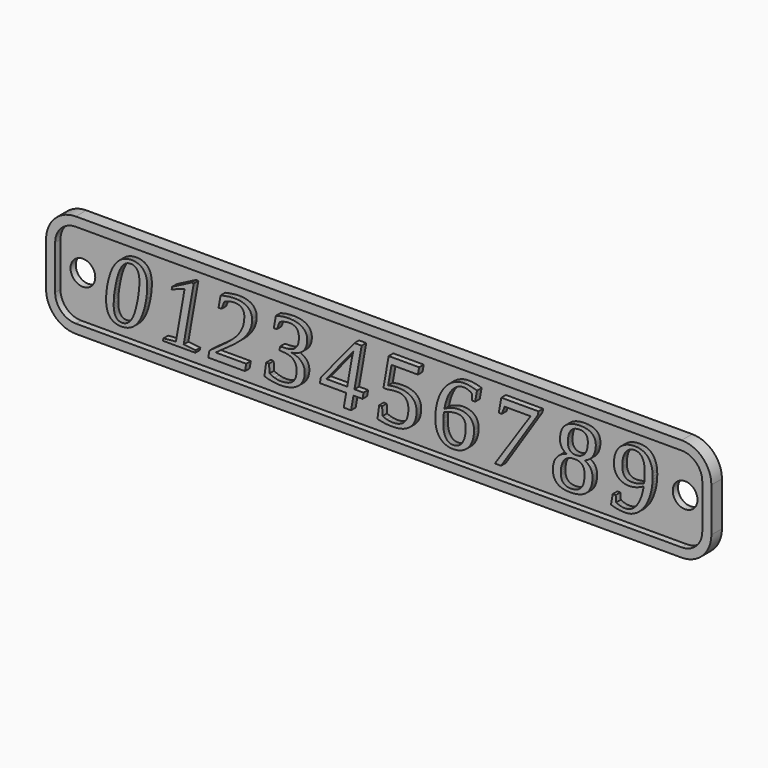
from build123d import *

# Parameters (mm, degrees)
F0_R     = 3
F1_DEPTH = 1.6
F2_DEPTH = 3.2
F3_DEPTH = 3


with BuildPart() as f1:
    # F0 (on Front) → F1 (new body)
    with BuildSketch(Plane.XZ):
        with BuildLine():
            Line((80.6455835819, -5.3311948478), (80.6455835819, 5.3311948478))
            ThreePointArc((80.6455835819, 5.3311948478), (78.5367524065, 10.4223636724), (73.4455835819, 12.5311948478))
            Line((73.4455835819, 12.5311948478), (-73.4455835819, 12.5311948478))
            ThreePointArc((-73.4455835819, 12.5311948478), (-78.5367524065, 10.4223636724), (-80.6455835819, 5.3311948478))
            Line((-80.6455835819, 5.3311948478), (-80.6455835819, -5.3311948478))
            ThreePointArc((-80.6455835819, -5.3311948478), (-78.5367524065, -10.4223636724), (-73.4455835819, -12.5311948478))
            Line((-73.4455835819, -12.5311948478), (73.4455835819, -12.5311948478))
            ThreePointArc((73.4455835819, -12.5311948478), (78.5367524065, -10.4223636724), (80.6455835819, -5.3311948478))
        make_face()
        with BuildLine():
            ThreePointArc((78.4455835819, -5.3311948478), (76.9811174879, -8.8667287538), (73.4455835819, -10.3311948478))
            Line((73.4455835819, -10.3311948478), (-73.4455835819, -10.3311948478))
            ThreePointArc((-73.4455835819, -10.3311948478), (-76.9811174879, -8.8667287538), (-78.4455835819, -5.3311948478))
            Line((-78.4455835819, -5.3311948478), (-78.4455835819, 5.3311948478))
            ThreePointArc((-78.4455835819, 5.3311948478), (-76.9811174879, 8.8667287538), (-73.4455835819, 10.3311948478))
            Line((-73.4455835819, 10.3311948478), (73.4455835819, 10.3311948478))
            ThreePointArc((73.4455835819, 10.3311948478), (76.9811174879, 8.8667287538), (78.4455835819, 5.3311948478))
            Line((78.4455835819, 5.3311948478), (78.4455835819, -5.3311948478))
        make_face(mode=Mode.SUBTRACT)
        with BuildLine():
            Line((-73.4455835819, -10.3311948478), (73.4455835819, -10.3311948478))
            ThreePointArc((73.4455835819, -10.3311948478), (76.9811174879, -8.8667287538), (78.4455835819, -5.3311948478))
            Line((78.4455835819, -5.3311948478), (78.4455835819, 5.3311948478))
            ThreePointArc((78.4455835819, 5.3311948478), (76.9811174879, 8.8667287538), (73.4455835819, 10.3311948478))
            Line((73.4455835819, 10.3311948478), (-73.4455835819, 10.3311948478))
            ThreePointArc((-73.4455835819, 10.3311948478), (-76.9811174879, 8.8667287538), (-78.4455835819, 5.3311948478))
            Line((-78.4455835819, 5.3311948478), (-78.4455835819, -5.3311948478))
            ThreePointArc((-78.4455835819, -5.3311948478), (-76.9811174879, -8.8667287538), (-73.4455835819, -10.3311948478))
        make_face()
        with Locations((-73, 0)):
            Circle(F0_R, mode=Mode.SUBTRACT)
        Polygon((-56.4955, 0.445), (-56.5613, 0.0543), (-56.7363, -0.8317), (-56.9357, -1.666), (-57.1596, -2.4489), (-57.4079, -3.1802), (-57.6772, -3.8578), (-57.8225, -4.1758), (-57.975, -4.4799), (-58.1346, -4.7701), (-58.3013, -5.0463), (-58.4751, -5.3087), (-58.6561, -5.5571), (-58.8443, -5.7888), (-59.04, -6.0062), (-59.2432, -6.2094), (-59.4538, -6.3983), (-59.6719, -6.573), (-59.8975, -6.7334), (-60.1305, -6.8796), (-60.371, -7.0116), (-60.6165, -7.126), (-60.8702, -7.2252), (-61.1321, -7.3092), (-61.4021, -7.3779), (-61.6802, -7.4313), (-61.9665, -7.4695), (-62.2609, -7.4923), (-62.5634, -7.5), (-62.7853, -7.4956), (-63.0005, -7.4825), (-63.2089, -7.4607), (-63.4107, -7.4301), (-63.6058, -7.3908), (-63.7942, -7.3428), (-63.9758, -7.286), (-64.1508, -7.2205), (-64.3191, -7.1463), (-64.4807, -7.0633), (-64.6355, -6.9716), (-64.7837, -6.8711), (-64.9252, -6.762), (-65.06, -6.6441), (-65.1881, -6.5174), (-65.3095, -6.382), (-65.4238, -6.2364), (-65.5308, -6.0815), (-65.6304, -5.9175), (-65.7226, -5.7444), (-65.8074, -5.5621), (-65.8849, -5.3706), (-65.955, -5.17), (-66.0177, -4.9602), (-66.073, -4.7412), (-66.121, -4.5131), (-66.1615, -4.2759), (-66.1947, -4.0295), (-66.2205, -3.7739), (-66.2501, -3.2353), (-66.2537, -2.9522), (-66.2497, -2.6239), (-66.2375, -2.2793), (-66.2171, -1.9184), (-66.1886, -1.5412), (-66.1513, -1.1484), (-66.0482, -0.3507), (-65.9824, 0.0543), (-65.8074, 0.9294), (-65.6079, 1.7529), (-65.3841, 2.5249), (-65.1358, 3.2453), (-64.8617, 3.9122), (-64.7145, 4.2247), (-64.5605, 4.5234), (-64.3998, 4.8081), (-64.2322, 5.0789), (-64.0579, 5.3359), (-63.8768, 5.5789), (-63.6888, 5.8078), (-63.4942, 6.0225), (-63.2927, 6.223), (-63.0844, 6.4092), (-62.8694, 6.5812), (-62.6476, 6.7389), (-62.419, 6.8824), (-62.1836, 7.0116), (-61.941, 7.1261), (-61.6911, 7.2253), (-61.4336, 7.3092), (-61.1687, 7.3779), (-60.8964, 7.4313), (-60.6165, 7.4695), (-60.3292, 7.4924), (-60.0345, 7.5), (-59.8125, 7.4958), (-59.597, 7.4831), (-59.3878, 7.4619), (-59.1852, 7.4322), (-58.989, 7.394), (-58.7992, 7.3474), (-58.6159, 7.2923), (-58.439, 7.2287), (-58.2685, 7.1566), (-58.1046, 7.076), (-57.947, 6.987), (-57.7959, 6.8895), (-57.6512, 6.7835), (-57.513, 6.669), (-57.3812, 6.5461), (-57.2559, 6.4146), (-57.1376, 6.2743), (-57.027, 6.1245), (-56.9239, 5.9653), (-56.8285, 5.7967), (-56.7408, 5.6186), (-56.6607, 5.4312), (-56.5882, 5.2343), (-56.5233, 5.0281), (-56.466, 4.8124), (-56.4164, 4.5873), (-56.3745, 4.3528), (-56.3401, 4.1089), (-56.3134, 3.8556), (-56.2943, 3.5928), (-56.2829, 3.3207), (-56.2791, 3.0391), (-56.2838, 2.7142), (-56.2981, 2.3689), (-56.3218, 2.0032), (-56.3551, 1.6172), (-56.3924, 1.2265), align=None, mode=Mode.SUBTRACT)
        Polygon((-23.3545, -7.4817), (-23.9623, -7.5), (-24.2296, -7.4966), (-24.7723, -7.4695), (-25.0477, -7.4457), (-25.3177, -7.4159), (-25.8495, -7.3399), (-26.1114, -7.2938), (-26.3631, -7.2483), (-26.846, -7.1452), (-27.0774, -7.0875), (-27.2938, -7.0272), (-27.498, -6.9654), (-27.6899, -6.9023), (-27.8697, -6.8379), (-27.4681, -3.7771), (-26.7518, -3.7771), (-26.6215, -5.8176), (-26.5708, -5.8555), (-26.5164, -5.8929), (-26.4582, -5.9301), (-26.3963, -5.9669), (-26.3307, -6.0033), (-26.2613, -6.0395), (-26.1882, -6.0752), (-26.1114, -6.1107), (-25.9506, -6.1751), (-25.6087, -6.2999), (-25.4276, -6.3603), (-25.2424, -6.4119), (-24.8679, -6.4987), (-24.6787, -6.534), (-24.4874, -6.5625), (-24.3042, -6.5828), (-24.1292, -6.595), (-23.9623, -6.5991), (-23.704, -6.5957), (-23.4556, -6.5855), (-23.217, -6.5686), (-22.9882, -6.5448), (-22.7692, -6.5143), (-22.5601, -6.477), (-22.3609, -6.4329), (-22.1714, -6.382), (-21.9912, -6.3218), (-21.8194, -6.2552), (-21.6561, -6.1821), (-21.5012, -6.1025), (-21.3549, -6.0166), (-21.217, -5.9241), (-21.0876, -5.8253), (-20.9667, -5.7199), (-20.8539, -5.6053), (-20.7489, -5.4839), (-20.6517, -5.3557), (-20.5624, -5.2207), (-20.4808, -5.0789), (-20.407, -4.9303), (-20.341, -4.775), (-20.2829, -4.6129), (-20.232, -4.4438), (-20.1879, -4.2676), (-20.1506, -4.0842), (-20.1201, -3.8938), (-20.0963, -3.6962), (-20.0794, -3.4915), (-20.0692, -3.2797), (-20.0658, -3.0608), (-20.0687, -2.8951), (-20.0775, -2.7345), (-20.0921, -2.5789), (-20.1126, -2.4285), (-20.1389, -2.2832), (-20.1711, -2.1429), (-20.2091, -2.0078), (-20.253, -1.8777), (-20.3028, -1.7527), (-20.3583, -1.6328), (-20.4198, -1.518), (-20.4871, -1.4083), (-20.5602, -1.3036), (-20.6392, -1.2041), (-20.724, -1.1096), (-20.8147, -1.0202), (-20.9097, -0.9357), (-21.0101, -0.8557), (-21.1159, -0.7804), (-21.2272, -0.7095), (-21.3438, -0.6433), (-21.4659, -0.5817), (-21.5935, -0.5246), (-21.7264, -0.4721), (-21.8648, -0.4242), (-22.0086, -0.3809), (-22.1579, -0.3421), (-22.3125, -0.308), (-22.6382, -0.2533), (-22.9855, -0.2171), (-24.2337, -0.1302), (-24.0817, 0.7598), (-22.5079, 0.8575), (-22.303, 0.8741), (-22.1063, 0.8968), (-21.9177, 0.9257), (-21.7373, 0.9606), (-21.565, 1.0016), (-21.4008, 1.0488), (-21.2448, 1.102), (-21.0969, 1.1614), (-20.9567, 1.2265), (-20.8235, 1.2971), (-20.6975, 1.373), (-20.5786, 1.4544), (-20.4669, 1.5413), (-20.3622, 1.6335), (-20.2647, 1.7312), (-20.1743, 1.8343), (-20.088, 1.9425), (-20.0081, 2.0555), (-19.9347, 2.1732), (-19.8677, 2.2956), (-19.8072, 2.4228), (-19.7531, 2.5547), (-19.7054, 2.6914), (-19.6642, 2.8329), (-19.5977, 3.1334), (-19.5502, 3.4488), (-19.5217, 3.7792), (-19.5122, 4.1245), (-19.5145, 4.2714), (-19.5211, 4.4136), (-19.5321, 4.5512), (-19.5475, 4.6841), (-19.5674, 4.8124), (-19.5916, 4.936), (-19.6203, 5.0549), (-19.6533, 5.1692), (-19.6908, 5.2788), (-19.7327, 5.3837), (-19.779, 5.484), (-19.8297, 5.5796), (-19.8848, 5.6705), (-19.9444, 5.7568), (-20.0083, 5.8384), (-20.0766, 5.9154), (-20.1497, 5.989), (-20.2278, 6.0578), (-20.3108, 6.1219), (-20.3989, 6.1813), (-20.4919, 6.2359), (-20.59, 6.2858), (-20.6931, 6.3309), (-20.8011, 6.3712), (-20.9142, 6.4068), (-21.0323, 6.4377), (-21.1554, 6.4638), (-21.2835, 6.4852), (-21.4165, 6.5018), (-21.5546, 6.5137), (-21.6977, 6.5208), (-21.8458, 6.5232), (-22.0086, 6.5198), (-22.3342, 6.4927), (-22.4971, 6.4689), (-22.6585, 6.4445), (-22.9733, 6.3794), (-23.1266, 6.3387), (-23.2765, 6.2986), (-23.5641, 6.2064), (-23.7018, 6.1541), (-23.8334, 6.1046), (-23.9569, 6.0538), (-24.0722, 6.0015), (-24.1794, 5.9479), (-24.874, 4.1679), (-25.5904, 4.1679), (-25.102, 6.9682), (-24.9181, 7.0163), (-24.5545, 7.1086), (-24.3748, 7.1527), (-24.1889, 7.1948), (-23.809, 7.2707), (-23.615, 7.3047), (-23.4115, 7.3352), (-22.9882, 7.384), (-22.7684, 7.4023), (-22.535, 7.4166), (-22.2908, 7.4268), (-22.0358, 7.4329), (-21.7698, 7.4349), (-21.2692, 7.4207), (-21.0301, 7.4028), (-20.7984, 7.3779), (-20.5742, 7.3459), (-20.3575, 7.3067), (-20.1482, 7.2604), (-19.9464, 7.207), (-19.7497, 7.1496), (-19.5611, 7.0862), (-19.3806, 7.0167), (-19.2083, 6.9411), (-19.0442, 6.8593), (-18.8882, 6.7715), (-18.7403, 6.6775), (-18.6005, 6.5774), (-18.4689, 6.4742), (-18.3455, 6.3651), (-18.2301, 6.2503), (-18.123, 6.1297), (-18.0239, 6.0034), (-17.933, 5.8713), (-17.8503, 5.7334), (-17.7756, 5.5897), (-17.7095, 5.441), (-17.6522, 5.2879), (-17.6037, 5.1303), (-17.564, 4.9684), (-17.5331, 4.802), (-17.5111, 4.6312), (-17.4978, 4.456), (-17.4934, 4.2764), (-17.4972, 4.0766), (-17.5084, 3.8815), (-17.527, 3.691), (-17.5531, 3.5051), (-17.5867, 3.324), (-17.6278, 3.1475), (-17.6763, 2.9756), (-17.7322, 2.8085), (-17.7956, 2.6459), (-17.8665, 2.4881), (-17.9449, 2.3349), (-18.0307, 2.1864), (-18.124, 2.0425), (-18.2247, 1.9033), (-18.3329, 1.7688), (-18.4486, 1.639), (-18.5707, 1.5143), (-18.7009, 1.3954), (-18.8393, 1.2823), (-18.9858, 1.175), (-19.1405, 1.0734), (-19.3033, 0.9775), (-19.4743, 0.8875), (-19.6533, 0.8032), (-19.8406, 0.7247), (-20.0359, 0.6519), (-20.2395, 0.5849), (-20.4511, 0.5237), (-20.8988, 0.4186), (-21.3791, 0.3365), (-21.0135, 0.2727), (-20.6655, 0.19), (-20.3351, 0.0882), (-20.0224, -0.0325), (-19.8733, -0.1), (-19.73, -0.1723), (-19.5925, -0.2493), (-19.4607, -0.331), (-19.3347, -0.4175), (-19.2144, -0.5088), (-19.1, -0.6047), (-18.9913, -0.7055), (-18.8859, -0.8081), (-18.7871, -0.9151), (-18.6946, -1.0265), (-18.6087, -1.1423), (-18.5291, -1.2626), (-18.456, -1.3872), (-18.3894, -1.5163), (-18.3292, -1.6498), (-18.2758, -1.7873), (-18.2295, -1.9286), (-18.1903, -2.0736), (-18.1582, -2.2223), (-18.1333, -2.3748), (-18.1155, -2.531), (-18.1048, -2.6909), (-18.1012, -2.8545), (-18.1084, -3.1378), (-18.1297, -3.4122), (-18.1654, -3.6777), (-18.2152, -3.9345), (-18.2793, -4.1824), (-18.3577, -4.4216), (-18.4503, -4.6519), (-18.5571, -4.8733), (-18.6738, -5.086), (-18.8013, -5.2899), (-18.9397, -5.4849), (-19.0889, -5.6711), (-19.249, -5.8485), (-19.42, -6.0171), (-19.6018, -6.1768), (-19.7944, -6.3278), (-19.9969, -6.4697), (-20.2082, -6.6025), (-20.4284, -6.7261), (-20.6573, -6.8406), (-20.8951, -6.9459), (-21.1417, -7.0421), (-21.3971, -7.1291), (-21.6613, -7.2069), (-22.204, -7.3351), (-22.7684, -7.4267), align=None, mode=Mode.SUBTRACT)
        Polygon((4.269, 1.2245), (4.4997, 1.2265), (4.7826, 1.2226), (5.056, 1.2109), (5.3198, 1.1914), (5.5742, 1.1641), (5.8191, 1.129), (6.0545, 1.0861), (6.2804, 1.0354), (6.4968, 0.9769), (6.7039, 0.9136), (6.9018, 0.8432), (7.0905, 0.7657), (7.2701, 0.6811), (7.4406, 0.5894), (7.6019, 0.4905), (7.754, 0.3845), (7.8969, 0.2714), (8.0335, 0.1516), (8.1608, 0.0258), (8.279, -0.1061), (8.3881, -0.2442), (8.488, -0.3883), (8.5787, -0.5386), (8.6603, -0.695), (8.7327, -0.8574), (8.7988, -1.0257), (8.8561, -1.1993), (8.9047, -1.3784), (8.9443, -1.5629), (8.9752, -1.7529), (8.9973, -1.9482), (9.0105, -2.149), (9.0149, -2.3553), (9.0088, -2.6576), (8.9905, -2.9515), (8.9599, -3.237), (8.9172, -3.5139), (8.8623, -3.7824), (8.7951, -4.0424), (8.7157, -4.2939), (8.6241, -4.5369), (8.5232, -4.7711), (8.4105, -4.9961), (8.2858, -5.212), (8.1493, -5.4188), (8.0009, -5.6163), (7.8406, -5.8047), (7.6685, -5.984), (7.4845, -6.1541), (7.2915, -6.3147), (7.087, -6.4655), (6.8709, -6.6064), (6.6433, -6.7375), (6.4042, -6.8588), (6.1535, -6.9702), (5.8914, -7.0718), (5.6176, -7.1635), (5.3353, -7.2424), (5.0417, -7.3107), (4.7369, -7.3685), (4.421, -7.4159), (4.0939, -7.4527), (3.7555, -7.4789), (3.0453, -7.5), (2.5202, -7.4912), (2.0196, -7.4647), (1.5434, -7.4206), (1.0916, -7.3589), (0.6642, -7.2897), (0.2613, -7.2124), (-0.1173, -7.1269), (-0.4714, -7.0333), (-0.0589, -3.9725), (0.6574, -3.9725), (0.7877, -6.013), (0.8326, -6.0401), (0.8806, -6.0673), (0.9317, -6.0944), (0.9858, -6.1215), (1.0429, -6.1487), (1.1031, -6.1758), (1.2327, -6.2301), (1.3765, -6.283), (1.6804, -6.3807), (1.8405, -6.4254), (2.0047, -6.4621), (2.3411, -6.5272), (2.5134, -6.5557), (2.6905, -6.5747), (3.0324, -6.5964), (3.1972, -6.5991), (3.4604, -6.5944), (3.7128, -6.5801), (3.9543, -6.5564), (4.1849, -6.5231), (4.4047, -6.4804), (4.6137, -6.4282), (4.8117, -6.3664), (4.999, -6.2952), (5.1789, -6.2155), (5.3497, -6.1283), (5.5113, -6.0337), (5.6638, -5.9316), (5.8071, -5.822), (5.9412, -5.705), (6.0662, -5.5805), (6.182, -5.4486), (6.2919, -5.3095), (6.3937, -5.1637), (6.4873, -5.0111), (6.5728, -4.8516), (6.6501, -4.6854), (6.7193, -4.5125), (6.7804, -4.3327), (6.8333, -4.1461), (6.9187, -3.7513), (6.9798, -3.3375), (7.0164, -2.9047), (7.0286, -2.4529), (7.0205, -2.1748), (6.9961, -1.9048), (6.9554, -1.643), (6.8984, -1.3893), (6.8628, -1.2638), (6.8211, -1.1423), (6.7732, -1.025), (6.7193, -0.9117), (6.6593, -0.8025), (6.5931, -0.6973), (6.5209, -0.5963), (6.4425, -0.4993), (6.3577, -0.4068), (6.2662, -0.3195), (6.1678, -0.2372), (6.0626, -0.1601), (5.9507, -0.088), (5.832, -0.021), (5.7065, 0.0409), (5.5742, 0.0977), (5.4341, 0.1486), (5.2852, 0.1927), (5.1275, 0.23), (4.961, 0.2605), (4.7856, 0.2843), (4.6014, 0.3012), (4.4085, 0.3114), (4.2066, 0.3148), (3.8885, 0.3094), (3.2644, 0.2659), (2.9584, 0.228), (2.8133, 0.2062), (2.6762, 0.1845), (2.5474, 0.1628), (2.4266, 0.1411), (2.314, 0.1194), (2.2095, 0.0977), (2.1132, 0.076), (2.0681, 0.0651), (2.025, 0.0543), (0.983, 0.0543), (2.2529, 7.2721), (9.6336, 7.2721), (9.3405, 5.6115), (2.9367, 5.6115), (2.1227, 0.966), (2.2265, 0.9877), (2.4381, 1.0311), (2.546, 1.0528), (2.6627, 1.0739), (2.7848, 1.0935), (3.0453, 1.1288), (3.1904, 1.1492), (3.3438, 1.1668), (3.5052, 1.1817), (3.6748, 1.1939), (3.7637, 1.2016), (3.8566, 1.2082), (4.0547, 1.2184), align=None, mode=Mode.SUBTRACT)
        Polygon((18.1609, -7.4929), (17.8407, -7.5), (17.5943, -7.4947), (17.3543, -7.4789), (17.1208, -7.4527), (16.8937, -7.4159), (16.673, -7.3685), (16.4589, -7.3107), (16.2511, -7.2424), (16.0498, -7.1635), (15.8554, -7.0745), (15.6686, -6.9756), (15.4891, -6.8669), (15.3172, -6.7483), (15.1527, -6.62), (14.9956, -6.4818), (14.846, -6.3337), (14.7039, -6.1758), (14.5696, -6.0086), (14.4434, -5.8326), (14.3254, -5.6477), (14.2155, -5.454), (14.1137, -5.2515), (14.0201, -5.0402), (13.9347, -4.8201), (13.8573, -4.5911), (13.7886, -4.351), (13.7291, -4.1027), (13.6787, -3.8463), (13.6375, -3.5817), (13.6055, -3.309), (13.5689, -2.7392), (13.5643, -2.4421), (13.5792, -1.74), (13.624, -1.0555), (13.6986, -0.3887), (13.8031, 0.2605), (13.9394, 0.8941), (14.0988, 1.5033), (14.2813, 2.088), (14.4868, 2.6484), (14.7209, 3.1829), (14.978, 3.6903), (15.2581, 4.1706), (15.5614, 4.6238), (15.885, 5.0518), (16.2262, 5.4459), (16.585, 5.8061), (16.9615, 6.1324), (17.355, 6.4289), (17.7647, 6.6887), (18.1907, 6.9119), (18.633, 7.0984), (18.8594, 7.1773), (19.0882, 7.2456), (19.3193, 7.3035), (19.5529, 7.3508), (19.7888, 7.3876), (20.0271, 7.4139), (20.2677, 7.4296), (20.5107, 7.4349), (20.9456, 7.424), (21.3709, 7.3915), (21.7867, 7.3372), (22.1931, 7.2612), (22.5906, 7.171), (22.9691, 7.074), (23.3287, 6.9702), (23.6692, 6.8596), (23.2242, 4.3524), (22.5078, 4.3524), (22.3884, 5.8719), (22.1673, 6.011), (21.938, 6.1352), (21.7006, 6.2444), (21.455, 6.3387), (21.3299, 6.3819), (21.204, 6.4194), (21.0775, 6.4511), (20.9503, 6.477), (20.8224, 6.4972), (20.6939, 6.5116), (20.5647, 6.5203), (20.4347, 6.5232), (20.2039, 6.5155), (19.9782, 6.4927), (19.7576, 6.4545), (19.542, 6.4011), (19.3316, 6.3324), (19.1262, 6.2484), (18.9259, 6.1492), (18.7307, 6.0348), (18.5435, 5.9098), (18.3617, 5.7736), (18.1853, 5.6262), (18.0143, 5.4676), (17.8488, 5.2979), (17.6887, 5.1169), (17.5341, 4.9248), (17.3848, 4.7214), (17.1026, 4.2859), (16.8421, 3.8151), (16.6033, 3.3091), (16.3863, 2.7678), (16.1963, 2.1993), (16.0281, 1.6118), (15.8816, 1.0054), (15.7567, 0.3799), (15.9189, 0.4722), (16.0905, 0.5644), (16.2716, 0.6567), (16.4622, 0.7489), (16.6658, 0.8392), (17.0891, 1.0074), (17.3088, 1.0854), (17.5381, 1.158), (18.0048, 1.2828), (18.2423, 1.335), (18.4865, 1.3778), (18.7307, 1.4083), (18.9749, 1.4266), (19.2191, 1.4327), (19.6519, 1.4185), (19.8592, 1.4007), (20.0603, 1.3757), (20.2553, 1.3437), (20.4442, 1.3045), (20.6271, 1.2582), (20.8038, 1.2048), (20.974, 1.1446), (21.1375, 1.0779), (21.2942, 1.0049), (21.4442, 0.9253), (21.5873, 0.8393), (21.7236, 0.7469), (21.8532, 0.648), (21.976, 0.5427), (22.0918, 0.4338), (22.2005, 0.3189), (22.3021, 0.1978), (22.3966, 0.0706), (22.4839, -0.0627), (22.5641, -0.2021), (22.6372, -0.3476), (22.7032, -0.4993), (22.7617, -0.6536), (22.8124, -0.8127), (22.8553, -0.9765), (22.8904, -1.1451), (22.9177, -1.3184), (22.9372, -1.4964), (22.9489, -1.6793), (22.9528, -1.8668), (22.9332, -2.4245), (22.8741, -2.9685), (22.7758, -3.499), (22.6381, -4.0159), (22.5568, -4.2671), (22.4651, -4.5104), (22.3628, -4.746), (22.2501, -4.9737), (22.1268, -5.1937), (21.993, -5.4059), (21.8486, -5.6102), (21.6938, -5.8068), (21.5312, -5.9947), (21.358, -6.1731), (21.1743, -6.342), (20.9802, -6.5014), (20.7755, -6.6513), (20.5602, -6.7918), (20.3345, -6.9227), (20.0983, -7.0441), (19.8541, -7.151), (19.599, -7.2436), (19.3331, -7.3219), (19.0563, -7.386), (18.7687, -7.4359), (18.4702, -7.4715), align=None, mode=Mode.SUBTRACT)
        Polygon((30.3676, 5.6115), (29.673, 3.8314), (28.9566, 3.8314), (29.5645, 7.2721), (38.5731, 7.2721), (38.4212, 6.4363), (29.5102, -7.2829), (28.0015, -7.2829), (36.652, 5.6115), align=None, mode=Mode.SUBTRACT)
        Polygon((52.4641, 4.7433), (52.4677, 4.5695), (52.4534, 4.1462), (52.4356, 3.9427), (52.4107, 3.7446), (52.3786, 3.5519), (52.3395, 3.3647), (52.2932, 3.1829), (52.2397, 3.0065), (52.1156, 2.6748), (51.9711, 2.3634), (51.8063, 2.0724), (51.7162, 1.9345), (51.6211, 1.8018), (51.423, 1.5521), (51.2086, 1.3242), (51.0953, 1.2184), (50.978, 1.118), (50.8566, 1.023), (50.7311, 0.9335), (50.4774, 0.7761), (50.2155, 0.6404), (49.9455, 0.5264), (49.6674, 0.4342), (49.8945, 0.346), (50.109, 0.2442), (50.311, 0.1289), (50.5004, 0), (50.6773, -0.1424), (50.8416, -0.2985), (50.9934, -0.468), (51.1327, -0.6512), (51.1971, -0.7462), (51.3134, -0.9446), (51.4131, -1.1543), (51.4962, -1.3751), (51.5627, -1.6071), (51.6126, -1.8503), (51.6458, -2.1046), (51.6624, -2.3702), (51.6645, -2.5072), (51.6594, -2.8042), (51.6441, -3.0926), (51.6187, -3.3726), (51.5831, -3.6442), (51.5373, -3.9072), (51.4813, -4.1617), (51.4152, -4.4078), (51.3389, -4.6454), (51.252, -4.8742), (51.1544, -5.0938), (51.0458, -5.3043), (50.9264, -5.5056), (50.7962, -5.6977), (50.6551, -5.8807), (50.5031, -6.0546), (50.3403, -6.2192), (50.169, -6.3719), (49.9862, -6.515), (49.7919, -6.6486), (49.586, -6.7728), (49.3686, -6.8874), (49.1396, -6.9926), (48.8991, -7.0882), (48.6471, -7.1744), (48.3861, -7.2507), (48.1133, -7.3168), (47.8285, -7.3728), (47.5319, -7.4186), (47.2234, -7.4542), (46.903, -7.4796), (46.5708, -7.4949), (46.2267, -7.5), (45.7147, -7.4862), (45.4716, -7.4691), (45.237, -7.445), (45.011, -7.4141), (44.7935, -7.3763), (44.5846, -7.3317), (44.3843, -7.2802), (44.1925, -7.2218), (44.0093, -7.1566), (43.8347, -7.0844), (43.6686, -7.0054), (43.5111, -6.9196), (43.3622, -6.8269), (43.2218, -6.7273), (43.09, -6.6208), (42.9664, -6.5067), (42.8508, -6.3868), (42.7432, -6.2611), (42.6436, -6.1297), (42.5519, -5.9925), (42.4682, -5.8495), (42.3925, -5.7008), (42.3248, -5.5463), (42.265, -5.386), (42.2132, -5.22), (42.1693, -5.0482), (42.1335, -4.8706), (42.1056, -4.6873), (42.0856, -4.4982), (42.0737, -4.3034), (42.0697, -4.1027), (42.0833, -3.6555), (42.124, -3.231), (42.1918, -2.8293), (42.2359, -2.6369), (42.2868, -2.4502), (42.3444, -2.2692), (42.4089, -2.0939), (42.4801, -1.9243), (42.5581, -1.7603), (42.6429, -1.6021), (42.7345, -1.4495), (42.8329, -1.3026), (42.938, -1.1613), (43.1666, -0.8919), (43.4183, -0.6424), (43.693, -0.4129), (43.9908, -0.2035), (44.3117, -0.0141), (44.6556, 0.1554), (45.0226, 0.3048), (45.4127, 0.4342), (45.2426, 0.5154), (45.0796, 0.6072), (44.9237, 0.7094), (44.775, 0.8222), (44.6334, 0.9455), (44.4989, 1.0793), (44.3716, 1.2236), (44.2513, 1.3785), (44.1961, 1.4612), (44.1445, 1.5465), (44.0964, 1.6345), (44.0519, 1.7251), (43.9735, 1.9142), (43.9094, 2.1138), (43.8596, 2.3239), (43.824, 2.5446), (43.8026, 2.7757), (43.7955, 3.0174), (43.8, 3.2747), (43.8138, 3.5255), (43.8367, 3.7699), (43.8687, 4.0078), (43.9099, 4.2393), (43.9603, 4.4643), (44.0198, 4.6829), (44.0885, 4.8951), (44.1667, 5.1), (44.2547, 5.2967), (44.3526, 5.4853), (44.4603, 5.6657), (44.5778, 5.838), (44.7051, 6.0022), (44.8423, 6.1582), (44.9894, 6.3061), (45.1463, 6.4457), (45.313, 6.5768), (45.4895, 6.6994), (45.6759, 6.8135), (45.8721, 6.9192), (46.0782, 7.0163), (46.294, 7.105), (46.5198, 7.1853), (46.7582, 7.259), (47.0068, 7.323), (47.2656, 7.3771), (47.5346, 7.4213), (47.8138, 7.4558), (48.1031, 7.4804), (48.4026, 7.4951), (48.7122, 7.5), (49.1768, 7.4882), (49.3972, 7.4733), (49.6097, 7.4525), (49.8144, 7.4258), (50.0111, 7.3932), (50.2, 7.3546), (50.381, 7.3101), (50.5541, 7.2596), (50.7194, 7.2032), (50.8767, 7.1409), (51.0261, 7.0727), (51.1677, 6.9985), (51.3014, 6.9183), (51.4272, 6.8323), (51.5451, 6.7403), (51.6568, 6.6427), (51.7613, 6.5401), (51.8586, 6.4324), (51.9487, 6.3197), (52.0316, 6.2018), (52.1073, 6.0789), (52.1758, 5.9508), (52.237, 5.8177), (52.2911, 5.6795), (52.3379, 5.5362), (52.3776, 5.3878), (52.41, 5.2343), (52.4352, 5.0757), (52.4533, 4.9121), align=None, mode=Mode.SUBTRACT)
        Polygon((61.6671, 7.4286), (61.9773, 7.4349), (62.2237, 7.4298), (62.4636, 7.4146), (62.6972, 7.3891), (62.9243, 7.3535), (63.1449, 7.3077), (63.3591, 7.2517), (63.5668, 7.1856), (63.7681, 7.1093), (63.9625, 7.0255), (64.1494, 6.9316), (64.3288, 6.8274), (64.5008, 6.7131), (64.6653, 6.5886), (64.8223, 6.454), (64.9719, 6.3092), (65.114, 6.1541), (65.2483, 5.9917), (65.3745, 5.819), (65.4925, 5.6362), (65.6024, 5.4432), (65.7042, 5.2401), (65.7978, 5.0267), (65.8833, 4.8032), (65.9606, 4.5695), (66.0293, 4.3287), (66.0888, 4.0784), (66.1392, 3.8185), (66.1804, 3.5492), (66.2125, 3.2704), (66.2354, 2.9821), (66.2537, 2.377), (66.2394, 1.6898), (66.1967, 1.0176), (66.1255, 0.3602), (66.0257, -0.2822), (65.8989, -0.9022), (65.7463, -1.5032), (65.5678, -2.0853), (65.3637, -2.6483), (65.1412, -3.1842), (64.8969, -3.6957), (64.631, -4.1828), (64.3434, -4.6454), (64.0354, -5.0748), (63.7084, -5.473), (63.3625, -5.84), (62.9975, -6.1758), (62.6204, -6.4729), (62.2269, -6.7348), (61.8172, -6.9614), (61.3912, -7.1527), (61.1753, -7.2341), (60.9563, -7.3046), (60.7343, -7.3643), (60.5093, -7.4131), (60.2812, -7.4511), (60.05, -7.4783), (59.8158, -7.4946), (59.5786, -7.5), (59.0834, -7.4905), (58.6071, -7.462), (58.1499, -7.4145), (57.7117, -7.348), (57.2925, -7.2639), (56.8922, -7.1635), (56.511, -7.0468), (56.1488, -6.9139), (56.5721, -4.5152), (57.2884, -4.5152), (57.4078, -6.0347), (57.5031, -6.0883), (57.6045, -6.1405), (57.712, -6.1914), (57.8257, -6.2409), (57.9454, -6.2891), (58.0712, -6.3359), (58.2032, -6.3814), (58.3412, -6.4254), (58.6316, -6.4967), (58.9273, -6.5476), (59.2285, -6.5781), (59.5351, -6.5883), (59.7709, -6.5808), (60.0005, -6.5584), (60.224, -6.5211), (60.4414, -6.4689), (60.6528, -6.4017), (60.858, -6.3196), (61.0571, -6.2226), (61.2501, -6.1107), (61.4368, -5.9832), (61.6171, -5.8448), (61.7909, -5.6955), (61.9583, -5.5354), (62.1192, -5.3645), (62.2737, -5.1827), (62.4218, -4.99), (62.5634, -4.7865), (62.834, -4.3463), (63.0816, -3.8721), (63.3062, -3.364), (63.5077, -2.822), (63.6861, -2.2535), (63.8414, -1.666), (63.9737, -1.0596), (64.0829, -0.4341), (63.9201, -0.5271), (63.7464, -0.6214), (63.5619, -0.717), (63.3666, -0.814), (63.1671, -0.9042), (62.7438, -1.0725), (62.52, -1.1505), (62.29, -1.2231), (61.8178, -1.3479), (61.5757, -1.4001), (61.3315, -1.4429), (61.0872, -1.4734), (60.843, -1.4917), (60.5988, -1.4978), (60.3794, -1.4937), (60.166, -1.4815), (59.9588, -1.4612), (59.7577, -1.4327), (59.5626, -1.3961), (59.3737, -1.3513), (59.1909, -1.2984), (59.0142, -1.2373), (58.8439, -1.1688), (58.6804, -1.0935), (58.5237, -1.0114), (58.3738, -0.9226), (58.2307, -0.8269), (58.0943, -0.7245), (57.9647, -0.6153), (57.842, -0.4993), (57.7261, -0.3768), (57.6174, -0.2483), (57.5158, -0.1136), (57.4214, 0.0272), (57.334, 0.174), (57.2538, 0.327), (57.1807, 0.4861), (57.1147, 0.6513), (57.0562, 0.8246), (57.0055, 1.0026), (56.9626, 1.1855), (56.9275, 1.373), (56.9002, 1.5653), (56.8807, 1.7624), (56.869, 1.9642), (56.8651, 2.1708), (56.8855, 2.7203), (56.9465, 3.2507), (57.0483, 3.7622), (57.1144, 4.0109), (57.1907, 4.2547), (57.277, 4.4922), (57.3732, 4.7214), (57.4792, 4.9426), (57.595, 5.1556), (57.7207, 5.3605), (57.8562, 5.5572), (58.0015, 5.7458), (58.1567, 5.9262), (58.3217, 6.0978), (58.4966, 6.26), (58.6813, 6.4126), (58.8758, 6.5557), (59.0801, 6.6894), (59.2943, 6.8135), (59.5184, 6.9282), (59.7522, 7.0333), (59.9983, 7.1274), (60.2535, 7.209), (60.5179, 7.278), (60.7915, 7.3345), (61.0742, 7.3784), (61.3661, 7.4098), align=None, mode=Mode.SUBTRACT)
        with Locations((73, 0)):
            Circle(F0_R, mode=Mode.SUBTRACT)
        Polygon((-45.0112, 7.3915), (-47.4533, -6.4146), (-44.5227, -6.7076), (-44.6313, -7.2829), (-52.4569, -7.2829), (-52.3484, -6.7076), (-49.3201, -6.4146), (-47.2253, 5.4595), (-50.3513, 4.4067), (-50.2427, 4.9819), (-45.5756, 7.3915), align=None, mode=Mode.SUBTRACT)
        Polygon((-32.2888, -5.6114), (-32.5819, -7.2829), (-41.482, -7.2829), (-41.1998, -5.6874), (-40.6042, -5.2451), (-39.4537, -4.4093), (-38.8988, -4.0159), (-38.3609, -3.6285), (-37.3461, -2.8742), (-36.8692, -2.5072), (-36.4085, -2.1389), (-35.5565, -1.4062), (-35.1651, -1.0419), (-34.7995, -0.6682), (-34.4623, -0.2849), (-34.1537, 0.1079), (-33.8735, 0.5102), (-33.6178, 0.924), (-33.3932, 1.3513), (-33.1999, 1.7923), (-33.0378, 2.2468), (-32.9691, 2.4806), (-32.9095, 2.7209), (-32.8592, 2.9677), (-32.7859, 3.4805), (-32.7493, 4.0192), (-32.7447, 4.2981), (-32.7472, 4.4409), (-32.7545, 4.5786), (-32.7668, 4.7115), (-32.784, 4.8395), (-32.8062, 4.9625), (-32.8332, 5.0806), (-32.8652, 5.1938), (-32.9021, 5.3021), (-32.9439, 5.4055), (-32.9906, 5.5039), (-33.0422, 5.5975), (-33.0988, 5.6861), (-33.1603, 5.7698), (-33.2267, 5.8485), (-33.298, 5.9224), (-33.3742, 5.9913), (-33.4552, 6.0557), (-33.5408, 6.116), (-33.6309, 6.1721), (-33.7256, 6.224), (-33.8249, 6.2718), (-33.9288, 6.3154), (-34.0372, 6.3549), (-34.1503, 6.3902), (-34.2679, 6.4214), (-34.3901, 6.4484), (-34.5168, 6.4712), (-34.6482, 6.4899), (-34.7841, 6.5045), (-35.0697, 6.5211), (-35.2194, 6.5232), (-35.3829, 6.5198), (-35.7139, 6.4927), (-35.8815, 6.4689), (-36.0436, 6.4445), (-36.3638, 6.3794), (-36.5218, 6.3387), (-36.6718, 6.2986), (-36.9594, 6.2064), (-37.0971, 6.1541), (-37.2287, 6.1046), (-37.3522, 6.0538), (-37.4675, 6.0015), (-37.5747, 5.9479), (-38.2693, 4.1679), (-38.9857, 4.1679), (-38.4972, 6.9682), (-38.0665, 7.0618), (-37.2253, 7.2246), (-36.8149, 7.2938), (-36.3957, 7.3555), (-35.9629, 7.3996), (-35.5165, 7.4261), (-35.0566, 7.4349), (-34.5471, 7.4207), (-34.3051, 7.4028), (-34.0716, 7.3779), (-33.8465, 7.3459), (-33.63, 7.3067), (-33.4219, 7.2604), (-33.2223, 7.207), (-33.0284, 7.1496), (-32.8431, 7.0862), (-32.6662, 7.0167), (-32.4978, 6.9411), (-32.3379, 6.8593), (-32.1864, 6.7715), (-32.0434, 6.6775), (-31.909, 6.5774), (-31.7828, 6.4718), (-31.6647, 6.361), (-31.5548, 6.2452), (-31.4531, 6.1243), (-31.3595, 5.9983), (-31.274, 5.8672), (-31.1967, 5.731), (-31.1275, 5.5897), (-31.0664, 5.4437), (-31.0135, 5.2933), (-30.9687, 5.1385), (-30.9321, 4.9792), (-30.9036, 4.8156), (-30.8833, 4.6475), (-30.8711, 4.475), (-30.867, 4.2981), (-30.8873, 3.786), (-30.9128, 3.5365), (-30.9484, 3.2914), (-30.9942, 3.0508), (-31.0501, 2.8146), (-31.1163, 2.5827), (-31.1926, 2.3553), (-31.3717, 1.915), (-31.5833, 1.4843), (-31.8276, 1.063), (-32.1043, 0.6513), (-32.4069, 0.2476), (-32.7393, -0.1492), (-33.1015, -0.5393), (-33.4936, -0.9226), (-33.9115, -1.2977), (-34.8124, -2.052), (-35.2954, -2.4312), (-35.7926, -2.8077), (-36.84, -3.5729), (-37.3901, -3.9616), (-37.9532, -4.3578), (-39.1037, -5.1827), (-39.6912, -5.6114), align=None, mode=Mode.SUBTRACT)
        Polygon((-4.0873, -3.9399), (-6.2798, -3.9399), (-6.8768, -7.2829), (-8.6351, -7.2829), (-8.0381, -3.9399), (-14.4093, -3.9399), (-14.1922, -2.6375), (-6.041, 7.3481), (-4.3044, 7.3481), (-6.041, -2.5289), (-3.8485, -2.5289), align=None, mode=Mode.SUBTRACT)
        Polygon((-56.7363, -0.8317), (-56.5613, 0.0543), (-56.4955, 0.445), (-56.3924, 1.2265), (-56.3551, 1.6172), (-56.3218, 2.0032), (-56.2981, 2.3689), (-56.2838, 2.7142), (-56.2791, 3.0391), (-56.2829, 3.3207), (-56.2943, 3.5928), (-56.3134, 3.8556), (-56.3401, 4.1089), (-56.3745, 4.3528), (-56.4164, 4.5873), (-56.466, 4.8124), (-56.5233, 5.0281), (-56.5882, 5.2343), (-56.6607, 5.4312), (-56.7408, 5.6186), (-56.8285, 5.7967), (-56.9239, 5.9653), (-57.027, 6.1245), (-57.1376, 6.2743), (-57.2559, 6.4146), (-57.3812, 6.5461), (-57.513, 6.669), (-57.6512, 6.7835), (-57.7959, 6.8895), (-57.947, 6.987), (-58.1046, 7.076), (-58.2685, 7.1566), (-58.439, 7.2287), (-58.6159, 7.2923), (-58.7992, 7.3474), (-58.989, 7.394), (-59.1852, 7.4322), (-59.3878, 7.4619), (-59.597, 7.4831), (-59.8125, 7.4958), (-60.0345, 7.5), (-60.3292, 7.4924), (-60.6165, 7.4695), (-60.8964, 7.4313), (-61.1687, 7.3779), (-61.4336, 7.3092), (-61.6911, 7.2253), (-61.941, 7.1261), (-62.1836, 7.0116), (-62.419, 6.8824), (-62.6476, 6.7389), (-62.8694, 6.5812), (-63.0844, 6.4092), (-63.2927, 6.223), (-63.4942, 6.0225), (-63.6888, 5.8078), (-63.8768, 5.5789), (-64.0579, 5.3359), (-64.2322, 5.0789), (-64.3998, 4.8081), (-64.5605, 4.5234), (-64.7145, 4.2247), (-64.8617, 3.9122), (-65.1358, 3.2453), (-65.3841, 2.5249), (-65.6079, 1.7529), (-65.8074, 0.9294), (-65.9824, 0.0543), (-66.0482, -0.3507), (-66.1513, -1.1484), (-66.1886, -1.5412), (-66.2171, -1.9184), (-66.2375, -2.2793), (-66.2497, -2.6239), (-66.2537, -2.9522), (-66.2501, -3.2353), (-66.2205, -3.7739), (-66.1947, -4.0295), (-66.1615, -4.2759), (-66.121, -4.5131), (-66.073, -4.7412), (-66.0177, -4.9602), (-65.955, -5.17), (-65.8849, -5.3706), (-65.8074, -5.5621), (-65.7226, -5.7444), (-65.6304, -5.9175), (-65.5308, -6.0815), (-65.4238, -6.2364), (-65.3095, -6.382), (-65.1881, -6.5174), (-65.06, -6.6441), (-64.9252, -6.762), (-64.7837, -6.8711), (-64.6355, -6.9716), (-64.4807, -7.0633), (-64.3191, -7.1463), (-64.1508, -7.2205), (-63.9758, -7.286), (-63.7942, -7.3428), (-63.6058, -7.3908), (-63.4107, -7.4301), (-63.2089, -7.4607), (-63.0005, -7.4825), (-62.7853, -7.4956), (-62.5634, -7.5), (-62.2609, -7.4923), (-61.9665, -7.4695), (-61.6802, -7.4313), (-61.4021, -7.3779), (-61.1321, -7.3092), (-60.8702, -7.2252), (-60.6165, -7.126), (-60.371, -7.0116), (-60.1305, -6.8796), (-59.8975, -6.7334), (-59.6719, -6.573), (-59.4538, -6.3983), (-59.2432, -6.2094), (-59.04, -6.0062), (-58.8443, -5.7888), (-58.6561, -5.5571), (-58.4751, -5.3087), (-58.3013, -5.0463), (-58.1346, -4.7701), (-57.975, -4.4799), (-57.8225, -4.1758), (-57.6772, -3.8578), (-57.4079, -3.1802), (-57.1596, -2.4489), (-56.9357, -1.666), align=None)
        Polygon((-58.4946, 0.0753), (-58.5367, -0.1845), (-58.6818, -0.9436), (-58.8352, -1.6579), (-58.9966, -2.3274), (-59.1662, -2.9522), (-59.2523, -3.2475), (-59.4369, -3.8024), (-59.5352, -4.062), (-59.6377, -4.3098), (-59.7442, -4.5457), (-59.8547, -4.7697), (-59.9694, -4.9819), (-60.0857, -5.1793), (-60.2068, -5.3645), (-60.3326, -5.5375), (-60.4632, -5.6982), (-60.5986, -5.8468), (-60.7386, -5.9832), (-60.8835, -6.1073), (-61.0331, -6.2192), (-61.1879, -6.3184), (-61.3485, -6.4044), (-61.5149, -6.4772), (-61.687, -6.5367), (-61.8649, -6.583), (-62.0486, -6.6161), (-62.238, -6.6359), (-62.4332, -6.6425), (-62.5611, -6.6391), (-62.6842, -6.629), (-62.8026, -6.612), (-62.9162, -6.5883), (-63.0251, -6.5577), (-63.1292, -6.5204), (-63.2286, -6.4763), (-63.3232, -6.4254), (-63.4136, -6.3658), (-63.5003, -6.3006), (-63.5832, -6.2301), (-63.6624, -6.1541), (-63.7379, -6.0727), (-63.8096, -5.9859), (-63.8776, -5.8936), (-63.9419, -5.7959), (-63.9997, -5.6903), (-64.0538, -5.5795), (-64.1042, -5.4637), (-64.1508, -5.3428), (-64.1937, -5.2168), (-64.2329, -5.0857), (-64.2683, -4.9495), (-64.3001, -4.8082), (-64.3475, -4.5131), (-64.3815, -4.2031), (-64.4018, -3.8782), (-64.4086, -3.5383), (-64.4052, -3.1476), (-64.3781, -2.3336), (-64.3543, -1.9103), (-64.3136, -1.4652), (-64.2566, -0.9877), (-64.1834, -0.4775), (-64.0938, 0.0651), (-63.9541, 0.8256), (-63.8062, 1.544), (-63.6502, 2.2203), (-63.486, 2.8546), (-63.3975, 3.1551), (-63.2103, 3.7195), (-63.1116, 3.9834), (-63.0095, 4.2351), (-62.904, 4.4745), (-62.7951, 4.7018), (-62.6828, 4.9168), (-62.5667, 5.1195), (-62.4461, 5.3096), (-62.3211, 5.4871), (-62.1917, 5.6522), (-62.0579, 5.8046), (-61.9197, 5.9445), (-61.777, 6.0719), (-61.63, 6.1867), (-61.4776, 6.291), (-61.3186, 6.3814), (-61.1533, 6.4579), (-60.9815, 6.5205), (-60.8033, 6.5691), (-60.6186, 6.6039), (-60.4274, 6.6248), (-60.2299, 6.6317), (-60.0993, 6.6283), (-59.9734, 6.6181), (-59.8524, 6.6012), (-59.736, 6.5774), (-59.6244, 6.5469), (-59.5176, 6.5096), (-59.4155, 6.4655), (-59.3181, 6.4146), (-59.2227, 6.3599), (-59.1316, 6.2986), (-59.0449, 6.231), (-58.9627, 6.1569), (-58.8848, 6.0763), (-58.8114, 5.9893), (-58.7424, 5.8959), (-58.6778, 5.796), (-58.6149, 5.6927), (-58.5563, 5.5836), (-58.5022, 5.4688), (-58.4526, 5.3483), (-58.4073, 5.2219), (-58.3664, 5.0898), (-58.3299, 4.9519), (-58.2979, 4.8083), (-58.2457, 4.5057), (-58.2083, 4.1842), (-58.186, 3.8436), (-58.1785, 3.4841), (-58.1799, 3.3152), (-58.1839, 3.1341), (-58.1907, 2.9407), (-58.2002, 2.7352), (-58.2124, 2.5249), (-58.245, 2.0799), (-58.2653, 1.8452), (-58.2891, 1.6037), (-58.3488, 1.1044), (-58.3847, 0.8466), (-58.4186, 0.5909), align=None, mode=Mode.SUBTRACT)
        Polygon((52.4534, 4.1462), (52.4677, 4.5695), (52.4641, 4.7433), (52.4533, 4.9121), (52.4352, 5.0757), (52.41, 5.2343), (52.3776, 5.3878), (52.3379, 5.5362), (52.2911, 5.6795), (52.237, 5.8177), (52.1758, 5.9508), (52.1073, 6.0789), (52.0316, 6.2018), (51.9487, 6.3197), (51.8586, 6.4324), (51.7613, 6.5401), (51.6568, 6.6427), (51.5451, 6.7403), (51.4272, 6.8323), (51.3014, 6.9183), (51.1677, 6.9985), (51.0261, 7.0727), (50.8767, 7.1409), (50.7194, 7.2032), (50.5541, 7.2596), (50.381, 7.3101), (50.2, 7.3546), (50.0111, 7.3932), (49.8144, 7.4258), (49.6097, 7.4525), (49.3972, 7.4733), (49.1768, 7.4882), (48.7122, 7.5), (48.4026, 7.4951), (48.1031, 7.4804), (47.8138, 7.4558), (47.5346, 7.4213), (47.2656, 7.3771), (47.0068, 7.323), (46.7582, 7.259), (46.5198, 7.1853), (46.294, 7.105), (46.0782, 7.0163), (45.8721, 6.9192), (45.6759, 6.8135), (45.4895, 6.6994), (45.313, 6.5768), (45.1463, 6.4457), (44.9894, 6.3061), (44.8423, 6.1582), (44.7051, 6.0022), (44.5778, 5.838), (44.4603, 5.6657), (44.3526, 5.4853), (44.2547, 5.2967), (44.1667, 5.1), (44.0885, 4.8951), (44.0198, 4.6829), (43.9603, 4.4643), (43.9099, 4.2393), (43.8687, 4.0078), (43.8367, 3.7699), (43.8138, 3.5255), (43.8, 3.2747), (43.7955, 3.0174), (43.8026, 2.7757), (43.824, 2.5446), (43.8596, 2.3239), (43.9094, 2.1138), (43.9735, 1.9142), (44.0519, 1.7251), (44.0964, 1.6345), (44.1445, 1.5465), (44.1961, 1.4612), (44.2513, 1.3785), (44.3716, 1.2236), (44.4989, 1.0793), (44.6334, 0.9455), (44.775, 0.8222), (44.9237, 0.7094), (45.0796, 0.6072), (45.2426, 0.5154), (45.4127, 0.4342), (45.0226, 0.3048), (44.6556, 0.1554), (44.3117, -0.0141), (43.9908, -0.2035), (43.693, -0.4129), (43.4183, -0.6424), (43.1666, -0.8919), (42.938, -1.1613), (42.8329, -1.3026), (42.7345, -1.4495), (42.6429, -1.6021), (42.5581, -1.7603), (42.4801, -1.9243), (42.4089, -2.0939), (42.3444, -2.2692), (42.2868, -2.4502), (42.2359, -2.6369), (42.1918, -2.8293), (42.124, -3.231), (42.0833, -3.6555), (42.0697, -4.1027), (42.0737, -4.3034), (42.0856, -4.4982), (42.1056, -4.6873), (42.1335, -4.8706), (42.1693, -5.0482), (42.2132, -5.22), (42.265, -5.386), (42.3248, -5.5463), (42.3925, -5.7008), (42.4682, -5.8495), (42.5519, -5.9925), (42.6436, -6.1297), (42.7432, -6.2611), (42.8508, -6.3868), (42.9664, -6.5067), (43.09, -6.6208), (43.2218, -6.7273), (43.3622, -6.8269), (43.5111, -6.9196), (43.6686, -7.0054), (43.8347, -7.0844), (44.0093, -7.1566), (44.1925, -7.2218), (44.3843, -7.2802), (44.5846, -7.3317), (44.7935, -7.3763), (45.011, -7.4141), (45.237, -7.445), (45.4716, -7.4691), (45.7147, -7.4862), (46.2267, -7.5), (46.5708, -7.4949), (46.903, -7.4796), (47.2234, -7.4542), (47.5319, -7.4186), (47.8285, -7.3728), (48.1133, -7.3168), (48.3861, -7.2507), (48.6471, -7.1744), (48.8991, -7.0882), (49.1396, -6.9926), (49.3686, -6.8874), (49.586, -6.7728), (49.7919, -6.6486), (49.9862, -6.515), (50.169, -6.3719), (50.3403, -6.2192), (50.5031, -6.0546), (50.6551, -5.8807), (50.7962, -5.6977), (50.9264, -5.5056), (51.0458, -5.3043), (51.1544, -5.0938), (51.252, -4.8742), (51.3389, -4.6454), (51.4152, -4.4078), (51.4813, -4.1617), (51.5373, -3.9072), (51.5831, -3.6442), (51.6187, -3.3726), (51.6441, -3.0926), (51.6594, -2.8042), (51.6645, -2.5072), (51.6624, -2.3702), (51.6458, -2.1046), (51.6126, -1.8503), (51.5627, -1.6071), (51.4962, -1.3751), (51.4131, -1.1543), (51.3134, -0.9446), (51.1971, -0.7462), (51.1327, -0.6512), (50.9934, -0.468), (50.8416, -0.2985), (50.6773, -0.1424), (50.5004, 0), (50.311, 0.1289), (50.109, 0.2442), (49.8945, 0.346), (49.6674, 0.4342), (49.9455, 0.5264), (50.2155, 0.6404), (50.4774, 0.7761), (50.7311, 0.9335), (50.8566, 1.023), (50.978, 1.118), (51.0953, 1.2184), (51.2086, 1.3242), (51.423, 1.5521), (51.6211, 1.8018), (51.7162, 1.9345), (51.8063, 2.0724), (51.9711, 2.3634), (52.1156, 2.6748), (52.2397, 3.0065), (52.2932, 3.1829), (52.3395, 3.3647), (52.3786, 3.5519), (52.4107, 3.7446), (52.4356, 3.9427), align=None)
        Polygon((46.6037, -6.6378), (46.357, -6.6425), (46.2048, -6.6398), (46.0578, -6.6317), (45.9159, -6.6181), (45.779, -6.5991), (45.6472, -6.5747), (45.5205, -6.5448), (45.3989, -6.5096), (45.2824, -6.4689), (45.1736, -6.4231), (45.0694, -6.3725), (44.97, -6.3172), (44.8754, -6.2572), (44.7855, -6.1924), (44.7004, -6.1229), (44.62, -6.0486), (44.5444, -5.9696), (44.476, -5.8861), (44.4121, -5.7986), (44.3526, -5.7071), (44.2974, -5.6114), (44.2467, -5.5117), (44.2004, -5.4079), (44.1586, -5.3), (44.1211, -5.1881), (44.0641, -4.948), (44.0234, -4.6943), (43.999, -4.427), (43.9908, -4.1461), (44.0017, -3.6957), (44.0342, -3.267), (44.0885, -2.86), (44.1645, -2.4747), (44.214, -2.2883), (44.2703, -2.109), (44.3334, -1.9369), (44.4033, -1.7719), (44.4799, -1.614), (44.5634, -1.4632), (44.6536, -1.3196), (44.7506, -1.183), (44.8549, -1.0513), (44.967, -0.9273), (45.0869, -0.8111), (45.2146, -0.7028), (45.3501, -0.6022), (45.4934, -0.5094), (45.6445, -0.4245), (45.8034, -0.3473), (45.9708, -0.2786), (46.1473, -0.2191), (46.3331, -0.1687), (46.5279, -0.1275), (46.7319, -0.0955), (46.9451, -0.0726), (47.1674, -0.0588), (47.3989, -0.0542), (47.556, -0.057), (47.7069, -0.0651), (47.8517, -0.0787), (47.9905, -0.0977), (48.1231, -0.1221), (48.2496, -0.1519), (48.37, -0.1872), (48.4843, -0.2279), (48.593, -0.2737), (48.6966, -0.3242), (48.7952, -0.3795), (48.8886, -0.4396), (48.977, -0.5043), (49.0602, -0.5739), (49.1384, -0.6482), (49.2115, -0.7272), (49.2795, -0.8077), (49.3424, -0.892), (49.4003, -0.98), (49.453, -1.0718), (49.5007, -1.1673), (49.5432, -1.2665), (49.5807, -1.3694), (49.6131, -1.4761), (49.6701, -1.6986), (49.7108, -1.932), (49.7352, -2.1762), (49.7434, -2.4312), (49.7339, -2.8885), (49.7054, -3.3267), (49.6579, -3.7459), (49.5914, -4.1461), (49.5522, -4.3354), (49.5053, -4.5179), (49.4505, -4.6936), (49.3879, -4.8625), (49.3175, -5.0246), (49.2393, -5.18), (49.1534, -5.3285), (49.0596, -5.4703), (48.9602, -5.605), (48.852, -5.7322), (48.735, -5.8519), (48.6091, -5.9642), (48.4745, -6.069), (48.331, -6.1663), (48.1787, -6.2562), (48.0176, -6.3386), (47.8492, -6.4098), (47.6696, -6.4716), (47.4788, -6.5238), (47.2768, -6.5665), (47.0637, -6.5998), (46.8393, -6.6235), align=None, mode=Mode.SUBTRACT)
        Polygon((47.7932, 0.9056), (47.5834, 0.9009), (47.4556, 0.9034), (47.3325, 0.9111), (47.2141, 0.9238), (47.1005, 0.9416), (46.9916, 0.9645), (46.8874, 0.9925), (46.7881, 1.0255), (46.6934, 1.0637), (46.6061, 1.1063), (46.5232, 1.1526), (46.4446, 1.2026), (46.3705, 1.2564), (46.3008, 1.3138), (46.2355, 1.3751), (46.1747, 1.44), (46.1182, 1.5087), (46.0658, 1.5806), (46.0171, 1.6552), (45.9722, 1.7326), (45.931, 1.8126), (45.8935, 1.8954), (45.8597, 1.9808), (45.8297, 2.069), (45.8034, 2.1599), (45.7607, 2.3533), (45.7302, 2.5534), (45.7118, 2.7603), (45.7057, 2.974), (45.7139, 3.3478), (45.7383, 3.7093), (45.779, 4.0587), (45.836, 4.3958), (45.8716, 4.5612), (45.9133, 4.7208), (45.9611, 4.8746), (46.0151, 5.0226), (46.0751, 5.1649), (46.1412, 5.3014), (46.2135, 5.4322), (46.2918, 5.5572), (46.3768, 5.6786), (46.4689, 5.7933), (46.5681, 5.9011), (46.6744, 6.0022), (46.7879, 6.0965), (46.9085, 6.184), (47.0362, 6.2647), (47.171, 6.3387), (47.3167, 6.4073), (47.4715, 6.4669), (47.6355, 6.5172), (47.8087, 6.5585), (47.991, 6.5905), (48.1824, 6.6134), (48.3831, 6.6271), (48.5929, 6.6317), (48.7233, 6.6295), (48.8486, 6.6229), (48.9688, 6.6119), (49.084, 6.5964), (49.1941, 6.5766), (49.299, 6.5523), (49.3989, 6.5237), (49.4937, 6.4906), (49.5863, 6.4533), (49.6742, 6.4119), (49.7573, 6.3665), (49.8356, 6.317), (49.9092, 6.2634), (49.9781, 6.2057), (50.0422, 6.144), (50.1015, 6.0782), (50.1565, 6.011), (50.2074, 5.9398), (50.2542, 5.8645), (50.2969, 5.7851), (50.3356, 5.7017), (50.3702, 5.6142), (50.4007, 5.5226), (50.4272, 5.4269), (50.4526, 5.3304), (50.4746, 5.2309), (50.5086, 5.0226), (50.5289, 4.8022), (50.5357, 4.5695), (50.5269, 4.2195), (50.5004, 3.8748), (50.4563, 3.5357), (50.3946, 3.2019), (50.3561, 3.0388), (50.3112, 2.8804), (50.2598, 2.7267), (50.2019, 2.5778), (50.1377, 2.4337), (50.0669, 2.2943), (49.9898, 2.1596), (49.9062, 2.0297), (49.8185, 1.9052), (49.7237, 1.7868), (49.6218, 1.6746), (49.5127, 1.5684), (49.3965, 1.4683), (49.2733, 1.3744), (49.1428, 1.2865), (49.0053, 1.2048), (48.8596, 1.1336), (48.7048, 1.0718), (48.5408, 1.0196), (48.3676, 0.9769), (48.1853, 0.9436), (47.9939, 0.9199), align=None, mode=Mode.SUBTRACT)
        Polygon((17.5943, -7.4947), (17.8407, -7.5), (18.1609, -7.4929), (18.4702, -7.4715), (18.7687, -7.4359), (19.0563, -7.386), (19.3331, -7.3219), (19.599, -7.2436), (19.8541, -7.151), (20.0983, -7.0441), (20.3345, -6.9227), (20.5602, -6.7918), (20.7755, -6.6513), (20.9802, -6.5014), (21.1743, -6.342), (21.358, -6.1731), (21.5312, -5.9947), (21.6938, -5.8068), (21.8486, -5.6102), (21.993, -5.4059), (22.1268, -5.1937), (22.2501, -4.9737), (22.3628, -4.746), (22.4651, -4.5104), (22.5568, -4.2671), (22.6381, -4.0159), (22.7758, -3.499), (22.8741, -2.9685), (22.9332, -2.4245), (22.9528, -1.8668), (22.9489, -1.6793), (22.9372, -1.4964), (22.9177, -1.3184), (22.8904, -1.1451), (22.8553, -0.9765), (22.8124, -0.8127), (22.7617, -0.6536), (22.7032, -0.4993), (22.6372, -0.3476), (22.5641, -0.2021), (22.4839, -0.0627), (22.3966, 0.0706), (22.3021, 0.1978), (22.2005, 0.3189), (22.0918, 0.4338), (21.976, 0.5427), (21.8532, 0.648), (21.7236, 0.7469), (21.5873, 0.8393), (21.4442, 0.9253), (21.2942, 1.0049), (21.1375, 1.0779), (20.974, 1.1446), (20.8038, 1.2048), (20.6271, 1.2582), (20.4442, 1.3045), (20.2553, 1.3437), (20.0603, 1.3757), (19.8592, 1.4007), (19.6519, 1.4185), (19.2191, 1.4327), (18.9749, 1.4266), (18.7307, 1.4083), (18.4865, 1.3778), (18.2423, 1.335), (18.0048, 1.2828), (17.5381, 1.158), (17.3088, 1.0854), (17.0891, 1.0074), (16.6658, 0.8392), (16.4622, 0.7489), (16.2716, 0.6567), (16.0905, 0.5644), (15.9189, 0.4722), (15.7567, 0.3799), (15.8816, 1.0054), (16.0281, 1.6118), (16.1963, 2.1993), (16.3863, 2.7678), (16.6033, 3.3091), (16.8421, 3.8151), (17.1026, 4.2859), (17.3848, 4.7214), (17.5341, 4.9248), (17.6887, 5.1169), (17.8488, 5.2979), (18.0143, 5.4676), (18.1853, 5.6262), (18.3617, 5.7736), (18.5435, 5.9098), (18.7307, 6.0348), (18.9259, 6.1492), (19.1262, 6.2484), (19.3316, 6.3324), (19.542, 6.4011), (19.7576, 6.4545), (19.9782, 6.4927), (20.2039, 6.5155), (20.4347, 6.5232), (20.5647, 6.5203), (20.6939, 6.5116), (20.8224, 6.4972), (20.9503, 6.477), (21.0775, 6.4511), (21.204, 6.4194), (21.3299, 6.3819), (21.455, 6.3387), (21.7006, 6.2444), (21.938, 6.1352), (22.1673, 6.011), (22.3884, 5.8719), (22.5078, 4.3524), (23.2242, 4.3524), (23.6692, 6.8596), (23.3287, 6.9702), (22.9691, 7.074), (22.5906, 7.171), (22.1931, 7.2612), (21.7867, 7.3372), (21.3709, 7.3915), (20.9456, 7.424), (20.5107, 7.4349), (20.2677, 7.4296), (20.0271, 7.4139), (19.7888, 7.3876), (19.5529, 7.3508), (19.3193, 7.3035), (19.0882, 7.2456), (18.8594, 7.1773), (18.633, 7.0984), (18.1907, 6.9119), (17.7647, 6.6887), (17.355, 6.4289), (16.9615, 6.1324), (16.585, 5.8061), (16.2262, 5.4459), (15.885, 5.0518), (15.5614, 4.6238), (15.2581, 4.1706), (14.978, 3.6903), (14.7209, 3.1829), (14.4868, 2.6484), (14.2813, 2.088), (14.0988, 1.5033), (13.9394, 0.8941), (13.8031, 0.2605), (13.6986, -0.3887), (13.624, -1.0555), (13.5792, -1.74), (13.5643, -2.4421), (13.5689, -2.7392), (13.6055, -3.309), (13.6375, -3.5817), (13.6787, -3.8463), (13.7291, -4.1027), (13.7886, -4.351), (13.8573, -4.5911), (13.9347, -4.8201), (14.0201, -5.0402), (14.1137, -5.2515), (14.2155, -5.454), (14.3254, -5.6477), (14.4434, -5.8326), (14.5696, -6.0086), (14.7039, -6.1758), (14.846, -6.3337), (14.9956, -6.4818), (15.1527, -6.62), (15.3172, -6.7483), (15.4891, -6.8669), (15.6686, -6.9756), (15.8554, -7.0745), (16.0498, -7.1635), (16.2511, -7.2424), (16.4589, -7.3107), (16.673, -7.3685), (16.8937, -7.4159), (17.1208, -7.4527), (17.3543, -7.4789), align=None)
        Polygon((15.4883, -3.075), (15.4854, -2.822), (15.4881, -2.4977), (15.5098, -1.8573), (15.5288, -1.5412), (15.5532, -1.2224), (15.6184, -0.5929), (15.6591, -0.2822), (15.8409, -0.2177), (16.2207, -0.0929), (16.4188, -0.0325), (16.6196, 0.0299), (17.0212, 0.1384), (17.222, 0.1845), (17.4221, 0.2307), (17.8183, 0.3066), (18.0143, 0.3365), (18.2077, 0.3602), (18.5821, 0.3874), (18.7633, 0.3908), (18.9007, 0.3884), (19.0334, 0.3814), (19.1615, 0.3698), (19.2849, 0.3535), (19.4037, 0.3325), (19.5178, 0.3068), (19.6272, 0.2765), (19.732, 0.2415), (19.8321, 0.2019), (19.9275, 0.1576), (20.0183, 0.1086), (20.1044, 0.055), (20.1858, -0.0033), (20.2626, -0.0663), (20.3347, -0.1339), (20.4022, -0.2062), (20.4666, -0.2818), (20.5268, -0.3621), (20.5829, -0.447), (20.6349, -0.5366), (20.6827, -0.6308), (20.7263, -0.7297), (20.7658, -0.8333), (20.8011, -0.9415), (20.8322, -1.0545), (20.8592, -1.172), (20.8821, -1.2943), (20.9008, -1.4211), (20.9153, -1.5527), (20.9257, -1.6889), (20.934, -1.9754), (20.9225, -2.4557), (20.8879, -2.9197), (20.8302, -3.3674), (20.7495, -3.7988), (20.6498, -4.2092), (20.5903, -4.4048), (20.5243, -4.5939), (20.4519, -4.7765), (20.373, -4.9527), (20.2877, -5.1225), (20.196, -5.2858), (20.1003, -5.4391), (19.9979, -5.5843), (19.8887, -5.7213), (19.7727, -5.8502), (19.6499, -5.9709), (19.5203, -6.0836), (19.384, -6.188), (19.2408, -6.2843), (19.0935, -6.3683), (18.939, -6.4411), (18.7773, -6.5026), (18.6086, -6.553), (18.4327, -6.5922), (18.2497, -6.6201), (18.0596, -6.6369), (17.8624, -6.6425), (17.736, -6.6393), (17.6121, -6.6296), (17.4905, -6.6135), (17.3713, -6.591), (17.2544, -6.562), (17.1399, -6.5265), (17.0278, -6.4846), (16.9181, -6.4363), (16.8114, -6.3783), (16.7085, -6.3128), (16.6093, -6.2399), (16.5138, -6.1595), (16.4221, -6.0717), (16.334, -5.9764), (16.2497, -5.8736), (16.1692, -5.7634), (16.0925, -5.6452), (16.02, -5.5185), (15.9514, -5.3833), (15.887, -5.2397), (15.8266, -5.0875), (15.7703, -4.9269), (15.7181, -4.7579), (15.6699, -4.5803), (15.6267, -4.3937), (15.5892, -4.1977), (15.5575, -3.9922), (15.5315, -3.7771), (15.5113, -3.5526), (15.4969, -3.3185), align=None, mode=Mode.SUBTRACT)
        Polygon((62.2237, 7.4298), (61.9773, 7.4349), (61.6671, 7.4286), (61.3661, 7.4098), (61.0742, 7.3784), (60.7915, 7.3345), (60.5179, 7.278), (60.2535, 7.209), (59.9983, 7.1274), (59.7522, 7.0333), (59.5184, 6.9282), (59.2943, 6.8135), (59.0801, 6.6894), (58.8758, 6.5557), (58.6813, 6.4126), (58.4966, 6.26), (58.3217, 6.0978), (58.1567, 5.9262), (58.0015, 5.7458), (57.8562, 5.5572), (57.7207, 5.3605), (57.595, 5.1556), (57.4792, 4.9426), (57.3732, 4.7214), (57.277, 4.4922), (57.1907, 4.2547), (57.1144, 4.0109), (57.0483, 3.7622), (56.9465, 3.2507), (56.8855, 2.7203), (56.8651, 2.1708), (56.869, 1.9642), (56.8807, 1.7624), (56.9002, 1.5653), (56.9275, 1.373), (56.9626, 1.1855), (57.0055, 1.0026), (57.0562, 0.8246), (57.1147, 0.6513), (57.1807, 0.4861), (57.2538, 0.327), (57.334, 0.174), (57.4214, 0.0272), (57.5158, -0.1136), (57.6174, -0.2483), (57.7261, -0.3768), (57.842, -0.4993), (57.9647, -0.6153), (58.0943, -0.7245), (58.2307, -0.8269), (58.3738, -0.9226), (58.5237, -1.0114), (58.6804, -1.0935), (58.8439, -1.1688), (59.0142, -1.2373), (59.1909, -1.2984), (59.3737, -1.3513), (59.5626, -1.3961), (59.7577, -1.4327), (59.9588, -1.4612), (60.166, -1.4815), (60.3794, -1.4937), (60.5988, -1.4978), (60.843, -1.4917), (61.0872, -1.4734), (61.3315, -1.4429), (61.5757, -1.4001), (61.8178, -1.3479), (62.29, -1.2231), (62.52, -1.1505), (62.7438, -1.0725), (63.1671, -0.9042), (63.3666, -0.814), (63.5619, -0.717), (63.7464, -0.6214), (63.9201, -0.5271), (64.0829, -0.4341), (63.9737, -1.0596), (63.8414, -1.666), (63.6861, -2.2535), (63.5077, -2.822), (63.3062, -3.364), (63.0816, -3.8721), (62.834, -4.3463), (62.5634, -4.7865), (62.4218, -4.99), (62.2737, -5.1827), (62.1192, -5.3645), (61.9583, -5.5354), (61.7909, -5.6955), (61.6171, -5.8448), (61.4368, -5.9832), (61.2501, -6.1107), (61.0571, -6.2226), (60.858, -6.3196), (60.6528, -6.4017), (60.4414, -6.4689), (60.224, -6.5211), (60.0005, -6.5584), (59.7709, -6.5808), (59.5351, -6.5883), (59.2285, -6.5781), (58.9273, -6.5476), (58.6316, -6.4967), (58.3412, -6.4254), (58.2032, -6.3814), (58.0712, -6.3359), (57.9454, -6.2891), (57.8257, -6.2409), (57.712, -6.1914), (57.6045, -6.1405), (57.5031, -6.0883), (57.4078, -6.0347), (57.2884, -4.5152), (56.5721, -4.5152), (56.1488, -6.9139), (56.511, -7.0468), (56.8922, -7.1635), (57.2925, -7.2639), (57.7117, -7.348), (58.1499, -7.4145), (58.6071, -7.462), (59.0834, -7.4905), (59.5786, -7.5), (59.8158, -7.4946), (60.05, -7.4783), (60.2812, -7.4511), (60.5093, -7.4131), (60.7343, -7.3643), (60.9563, -7.3046), (61.1753, -7.2341), (61.3912, -7.1527), (61.8172, -6.9614), (62.2269, -6.7348), (62.6204, -6.4729), (62.9975, -6.1758), (63.3625, -5.84), (63.7084, -5.473), (64.0354, -5.0748), (64.3434, -4.6454), (64.631, -4.1828), (64.8969, -3.6957), (65.1412, -3.1842), (65.3637, -2.6483), (65.5678, -2.0853), (65.7463, -1.5032), (65.8989, -0.9022), (66.0257, -0.2822), (66.1255, 0.3602), (66.1967, 1.0176), (66.2394, 1.6898), (66.2537, 2.377), (66.2354, 2.9821), (66.2125, 3.2704), (66.1804, 3.5492), (66.1392, 3.8185), (66.0888, 4.0784), (66.0293, 4.3287), (65.9606, 4.5695), (65.8833, 4.8032), (65.7978, 5.0267), (65.7042, 5.2401), (65.6024, 5.4432), (65.4925, 5.6362), (65.3745, 5.819), (65.2483, 5.9917), (65.114, 6.1541), (64.9719, 6.3092), (64.8223, 6.454), (64.6653, 6.5886), (64.5008, 6.7131), (64.3288, 6.8274), (64.1494, 6.9316), (63.9625, 7.0255), (63.7681, 7.1093), (63.5668, 7.1856), (63.3591, 7.2517), (63.1449, 7.3077), (62.9243, 7.3535), (62.6972, 7.3891), (62.4636, 7.4146), align=None)
        Polygon((64.3297, 3.0099), (64.3325, 2.7569), (64.3298, 2.432), (64.3081, 1.7862), (64.2891, 1.4653), (64.2701, 1.1465), (64.2159, 0.5169), (64.1806, 0.2062), (63.8346, 0.0665), (63.1183, -0.1723), (62.7479, -0.2713), (62.3673, -0.352), (61.9745, -0.4097), (61.5696, -0.4443), (61.1524, -0.4558), (61.0212, -0.4533), (60.8936, -0.4457), (60.7695, -0.4329), (60.649, -0.4151), (60.5321, -0.3922), (60.4187, -0.3643), (60.3089, -0.3312), (60.2027, -0.293), (60.1, -0.2498), (60.0008, -0.2015), (59.9053, -0.148), (59.8133, -0.0895), (59.7248, -0.0259), (59.64, 0.0428), (59.5586, 0.1165), (59.4809, 0.1954), (59.4086, 0.2809), (59.341, 0.3719), (59.278, 0.4685), (59.2197, 0.5705), (59.1661, 0.6781), (59.1171, 0.7912), (59.0728, 0.9098), (59.0332, 1.0339), (58.9982, 1.1635), (58.9679, 1.2986), (58.9422, 1.4392), (58.9212, 1.5854), (58.9049, 1.737), (58.8932, 1.8942), (58.8863, 2.0569), (58.8839, 2.2251), (58.8948, 2.6782), (58.9273, 3.1151), (58.9816, 3.5357), (59.0576, 3.94), (59.1066, 4.1374), (59.1614, 4.328), (59.2219, 4.5118), (59.2882, 4.6889), (59.3603, 4.8591), (59.4381, 5.0226), (59.5218, 5.1793), (59.6111, 5.3293), (59.7091, 5.4717), (59.8133, 5.606), (59.9235, 5.7322), (60.0399, 5.8502), (60.1623, 5.9601), (60.2908, 6.0619), (60.4255, 6.1555), (60.5663, 6.241), (60.7162, 6.3198), (60.8729, 6.3882), (61.0364, 6.446), (61.2066, 6.4933), (61.3837, 6.5301), (61.5675, 6.5564), (61.7581, 6.5722), (61.9556, 6.5774), (62.0794, 6.5741), (62.2011, 6.5639), (62.3209, 6.5469), (62.4386, 6.5232), (62.5542, 6.4927), (62.6678, 6.4553), (62.7794, 6.4112), (62.889, 6.3604), (62.9982, 6.3049), (63.1033, 6.2417), (63.2044, 6.1706), (63.3014, 6.0917), (63.3944, 6.0051), (63.4832, 5.9106), (63.568, 5.8084), (63.6488, 5.6983), (63.7254, 5.5801), (63.798, 5.4534), (63.8665, 5.3182), (63.931, 5.1746), (63.9913, 5.0225), (64.0476, 4.8619), (64.0999, 4.6928), (64.148, 4.5152), (64.1913, 4.3287), (64.2288, 4.1326), (64.2605, 3.9271), (64.2864, 3.712), (64.3066, 3.4875), (64.321, 3.2535), align=None, mode=Mode.SUBTRACT)
        Polygon((-6.8768, -7.2829), (-6.2798, -3.9399), (-4.0873, -3.9399), (-3.8485, -2.5289), (-6.041, -2.5289), (-4.3044, 7.3481), (-6.041, 7.3481), (-14.1922, -2.6375), (-14.4093, -3.9399), (-8.0381, -3.9399), (-8.6351, -7.2829), align=None)
        Polygon((-6.7397, 3.4895), (-6.7682, 3.343), (-7.7993, -2.5289), (-12.8464, -2.5289), (-6.3015, 5.5246), (-6.3497, 5.3191), (-6.4419, 4.9121), (-6.486, 4.7106), (-6.524, 4.5356), (-6.6, 4.1774), (-6.638, 3.9942), (-6.6746, 3.8151), (-6.7085, 3.6469), align=None, mode=Mode.SUBTRACT)
        Polygon((-58.6818, -0.9436), (-58.5367, -0.1845), (-58.4946, 0.0753), (-58.4186, 0.5909), (-58.3847, 0.8466), (-58.3488, 1.1044), (-58.2891, 1.6037), (-58.2653, 1.8452), (-58.245, 2.0799), (-58.2124, 2.5249), (-58.2002, 2.7352), (-58.1907, 2.9407), (-58.1839, 3.1341), (-58.1799, 3.3152), (-58.1785, 3.4841), (-58.186, 3.8436), (-58.2083, 4.1842), (-58.2457, 4.5057), (-58.2979, 4.8083), (-58.3299, 4.9519), (-58.3664, 5.0898), (-58.4073, 5.2219), (-58.4526, 5.3483), (-58.5022, 5.4688), (-58.5563, 5.5836), (-58.6149, 5.6927), (-58.6778, 5.796), (-58.7424, 5.8959), (-58.8114, 5.9893), (-58.8848, 6.0763), (-58.9627, 6.1569), (-59.0449, 6.231), (-59.1316, 6.2986), (-59.2227, 6.3599), (-59.3181, 6.4146), (-59.4155, 6.4655), (-59.5176, 6.5096), (-59.6244, 6.5469), (-59.736, 6.5774), (-59.8524, 6.6012), (-59.9734, 6.6181), (-60.0993, 6.6283), (-60.2299, 6.6317), (-60.4274, 6.6248), (-60.6186, 6.6039), (-60.8033, 6.5691), (-60.9815, 6.5205), (-61.1533, 6.4579), (-61.3186, 6.3814), (-61.4776, 6.291), (-61.63, 6.1867), (-61.777, 6.0719), (-61.9197, 5.9445), (-62.0579, 5.8046), (-62.1917, 5.6522), (-62.3211, 5.4871), (-62.4461, 5.3096), (-62.5667, 5.1195), (-62.6828, 4.9168), (-62.7951, 4.7018), (-62.904, 4.4745), (-63.0095, 4.2351), (-63.1116, 3.9834), (-63.2103, 3.7195), (-63.3975, 3.1551), (-63.486, 2.8546), (-63.6502, 2.2203), (-63.8062, 1.544), (-63.9541, 0.8256), (-64.0938, 0.0651), (-64.1834, -0.4775), (-64.2566, -0.9877), (-64.3136, -1.4652), (-64.3543, -1.9103), (-64.3781, -2.3336), (-64.4052, -3.1476), (-64.4086, -3.5383), (-64.4018, -3.8782), (-64.3815, -4.2031), (-64.3475, -4.5131), (-64.3001, -4.8082), (-64.2683, -4.9495), (-64.2329, -5.0857), (-64.1937, -5.2168), (-64.1508, -5.3428), (-64.1042, -5.4637), (-64.0538, -5.5795), (-63.9997, -5.6903), (-63.9419, -5.7959), (-63.8776, -5.8936), (-63.8096, -5.9859), (-63.7379, -6.0727), (-63.6624, -6.1541), (-63.5832, -6.2301), (-63.5003, -6.3006), (-63.4136, -6.3658), (-63.3232, -6.4254), (-63.2286, -6.4763), (-63.1292, -6.5204), (-63.0251, -6.5577), (-62.9162, -6.5883), (-62.8026, -6.612), (-62.6842, -6.629), (-62.5611, -6.6391), (-62.4332, -6.6425), (-62.238, -6.6359), (-62.0486, -6.6161), (-61.8649, -6.583), (-61.687, -6.5367), (-61.5149, -6.4772), (-61.3485, -6.4044), (-61.1879, -6.3184), (-61.0331, -6.2192), (-60.8835, -6.1073), (-60.7386, -5.9832), (-60.5986, -5.8468), (-60.4632, -5.6982), (-60.3326, -5.5375), (-60.2068, -5.3645), (-60.0857, -5.1793), (-59.9694, -4.9819), (-59.8547, -4.7697), (-59.7442, -4.5457), (-59.6377, -4.3098), (-59.5352, -4.062), (-59.4369, -3.8024), (-59.2523, -3.2475), (-59.1662, -2.9522), (-58.9966, -2.3274), (-58.8352, -1.6579), align=None)
        Polygon((4.7826, 1.2226), (4.4997, 1.2265), (4.269, 1.2245), (4.0547, 1.2184), (3.8566, 1.2082), (3.7637, 1.2016), (3.6748, 1.1939), (3.5052, 1.1817), (3.3438, 1.1668), (3.1904, 1.1492), (3.0453, 1.1288), (2.7848, 1.0935), (2.6627, 1.0739), (2.546, 1.0528), (2.4381, 1.0311), (2.2265, 0.9877), (2.1227, 0.966), (2.9367, 5.6115), (9.3405, 5.6115), (9.6336, 7.2721), (2.2529, 7.2721), (0.983, 0.0543), (2.025, 0.0543), (2.0681, 0.0651), (2.1132, 0.076), (2.2095, 0.0977), (2.314, 0.1194), (2.4266, 0.1411), (2.5474, 0.1628), (2.6762, 0.1845), (2.8133, 0.2062), (2.9584, 0.228), (3.2644, 0.2659), (3.8885, 0.3094), (4.2066, 0.3148), (4.4085, 0.3114), (4.6014, 0.3012), (4.7856, 0.2843), (4.961, 0.2605), (5.1275, 0.23), (5.2852, 0.1927), (5.4341, 0.1486), (5.5742, 0.0977), (5.7065, 0.0409), (5.832, -0.021), (5.9507, -0.088), (6.0626, -0.1601), (6.1678, -0.2372), (6.2662, -0.3195), (6.3577, -0.4068), (6.4425, -0.4993), (6.5209, -0.5963), (6.5931, -0.6973), (6.6593, -0.8025), (6.7193, -0.9117), (6.7732, -1.025), (6.8211, -1.1423), (6.8628, -1.2638), (6.8984, -1.3893), (6.9554, -1.643), (6.9961, -1.9048), (7.0205, -2.1748), (7.0286, -2.4529), (7.0164, -2.9047), (6.9798, -3.3375), (6.9187, -3.7513), (6.8333, -4.1461), (6.7804, -4.3327), (6.7193, -4.5125), (6.6501, -4.6854), (6.5728, -4.8516), (6.4873, -5.0111), (6.3937, -5.1637), (6.2919, -5.3095), (6.182, -5.4486), (6.0662, -5.5805), (5.9412, -5.705), (5.8071, -5.822), (5.6638, -5.9316), (5.5113, -6.0337), (5.3497, -6.1283), (5.1789, -6.2155), (4.999, -6.2952), (4.8117, -6.3664), (4.6137, -6.4282), (4.4047, -6.4804), (4.1849, -6.5231), (3.9543, -6.5564), (3.7128, -6.5801), (3.4604, -6.5944), (3.1972, -6.5991), (3.0324, -6.5964), (2.6905, -6.5747), (2.5134, -6.5557), (2.3411, -6.5272), (2.0047, -6.4621), (1.8405, -6.4254), (1.6804, -6.3807), (1.3765, -6.283), (1.2327, -6.2301), (1.1031, -6.1758), (1.0429, -6.1487), (0.9858, -6.1215), (0.9317, -6.0944), (0.8806, -6.0673), (0.8326, -6.0401), (0.7877, -6.013), (0.6574, -3.9725), (-0.0589, -3.9725), (-0.4714, -7.0333), (-0.1173, -7.1269), (0.2613, -7.2124), (0.6642, -7.2897), (1.0916, -7.3589), (1.5434, -7.4206), (2.0196, -7.4647), (2.5202, -7.4912), (3.0453, -7.5), (3.7555, -7.4789), (4.0939, -7.4527), (4.421, -7.4159), (4.7369, -7.3685), (5.0417, -7.3107), (5.3353, -7.2424), (5.6176, -7.1635), (5.8914, -7.0718), (6.1535, -6.9702), (6.4042, -6.8588), (6.6433, -6.7375), (6.8709, -6.6064), (7.087, -6.4655), (7.2915, -6.3147), (7.4845, -6.1541), (7.6685, -5.984), (7.8406, -5.8047), (8.0009, -5.6163), (8.1493, -5.4188), (8.2858, -5.212), (8.4105, -4.9961), (8.5232, -4.7711), (8.6241, -4.5369), (8.7157, -4.2939), (8.7951, -4.0424), (8.8623, -3.7824), (8.9172, -3.5139), (8.9599, -3.237), (8.9905, -2.9515), (9.0088, -2.6576), (9.0149, -2.3553), (9.0105, -2.149), (8.9973, -1.9482), (8.9752, -1.7529), (8.9443, -1.5629), (8.9047, -1.3784), (8.8561, -1.1993), (8.7988, -1.0257), (8.7327, -0.8574), (8.6603, -0.695), (8.5787, -0.5386), (8.488, -0.3883), (8.3881, -0.2442), (8.279, -0.1061), (8.1608, 0.0258), (8.0335, 0.1516), (7.8969, 0.2714), (7.754, 0.3845), (7.6019, 0.4905), (7.4406, 0.5894), (7.2701, 0.6811), (7.0905, 0.7657), (6.9018, 0.8432), (6.7039, 0.9136), (6.4968, 0.9769), (6.2804, 1.0354), (6.0545, 1.0861), (5.8191, 1.129), (5.5742, 1.1641), (5.3198, 1.1914), (5.056, 1.2109), align=None)
        Polygon((-24.2296, -7.4966), (-23.9623, -7.5), (-23.3545, -7.4817), (-22.7684, -7.4267), (-22.204, -7.3351), (-21.6613, -7.2069), (-21.3971, -7.1291), (-21.1417, -7.0421), (-20.8951, -6.9459), (-20.6573, -6.8406), (-20.4284, -6.7261), (-20.2082, -6.6025), (-19.9969, -6.4697), (-19.7944, -6.3278), (-19.6018, -6.1768), (-19.42, -6.0171), (-19.249, -5.8485), (-19.0889, -5.6711), (-18.9397, -5.4849), (-18.8013, -5.2899), (-18.6738, -5.086), (-18.5571, -4.8733), (-18.4503, -4.6519), (-18.3577, -4.4216), (-18.2793, -4.1824), (-18.2152, -3.9345), (-18.1654, -3.6777), (-18.1297, -3.4122), (-18.1084, -3.1378), (-18.1012, -2.8545), (-18.1048, -2.6909), (-18.1155, -2.531), (-18.1333, -2.3748), (-18.1582, -2.2223), (-18.1903, -2.0736), (-18.2295, -1.9286), (-18.2758, -1.7873), (-18.3292, -1.6498), (-18.3894, -1.5163), (-18.456, -1.3872), (-18.5291, -1.2626), (-18.6087, -1.1423), (-18.6946, -1.0265), (-18.7871, -0.9151), (-18.8859, -0.8081), (-18.9913, -0.7055), (-19.1, -0.6047), (-19.2144, -0.5088), (-19.3347, -0.4175), (-19.4607, -0.331), (-19.5925, -0.2493), (-19.73, -0.1723), (-19.8733, -0.1), (-20.0224, -0.0325), (-20.3351, 0.0882), (-20.6655, 0.19), (-21.0135, 0.2727), (-21.3791, 0.3365), (-20.8988, 0.4186), (-20.4511, 0.5237), (-20.2395, 0.5849), (-20.0359, 0.6519), (-19.8406, 0.7247), (-19.6533, 0.8032), (-19.4743, 0.8875), (-19.3033, 0.9775), (-19.1405, 1.0734), (-18.9858, 1.175), (-18.8393, 1.2823), (-18.7009, 1.3954), (-18.5707, 1.5143), (-18.4486, 1.639), (-18.3329, 1.7688), (-18.2247, 1.9033), (-18.124, 2.0425), (-18.0307, 2.1864), (-17.9449, 2.3349), (-17.8665, 2.4881), (-17.7956, 2.6459), (-17.7322, 2.8085), (-17.6763, 2.9756), (-17.6278, 3.1475), (-17.5867, 3.324), (-17.5531, 3.5051), (-17.527, 3.691), (-17.5084, 3.8815), (-17.4972, 4.0766), (-17.4934, 4.2764), (-17.4978, 4.456), (-17.5111, 4.6312), (-17.5331, 4.802), (-17.564, 4.9684), (-17.6037, 5.1303), (-17.6522, 5.2879), (-17.7095, 5.441), (-17.7756, 5.5897), (-17.8503, 5.7334), (-17.933, 5.8713), (-18.0239, 6.0034), (-18.123, 6.1297), (-18.2301, 6.2503), (-18.3455, 6.3651), (-18.4689, 6.4742), (-18.6005, 6.5774), (-18.7403, 6.6775), (-18.8882, 6.7715), (-19.0442, 6.8593), (-19.2083, 6.9411), (-19.3806, 7.0167), (-19.5611, 7.0862), (-19.7497, 7.1496), (-19.9464, 7.207), (-20.1482, 7.2604), (-20.3575, 7.3067), (-20.5742, 7.3459), (-20.7984, 7.3779), (-21.0301, 7.4028), (-21.2692, 7.4207), (-21.7698, 7.4349), (-22.0358, 7.4329), (-22.2908, 7.4268), (-22.535, 7.4166), (-22.7684, 7.4023), (-22.9882, 7.384), (-23.4115, 7.3352), (-23.615, 7.3047), (-23.809, 7.2707), (-24.1889, 7.1948), (-24.3748, 7.1527), (-24.5545, 7.1086), (-24.9181, 7.0163), (-25.102, 6.9682), (-25.5904, 4.1679), (-24.874, 4.1679), (-24.1794, 5.9479), (-24.0722, 6.0015), (-23.9569, 6.0538), (-23.8334, 6.1046), (-23.7018, 6.1541), (-23.5641, 6.2064), (-23.2765, 6.2986), (-23.1266, 6.3387), (-22.9733, 6.3794), (-22.6585, 6.4445), (-22.4971, 6.4689), (-22.3342, 6.4927), (-22.0086, 6.5198), (-21.8458, 6.5232), (-21.6977, 6.5208), (-21.5546, 6.5137), (-21.4165, 6.5018), (-21.2835, 6.4852), (-21.1554, 6.4638), (-21.0323, 6.4377), (-20.9142, 6.4068), (-20.8011, 6.3712), (-20.6931, 6.3309), (-20.59, 6.2858), (-20.4919, 6.2359), (-20.3989, 6.1813), (-20.3108, 6.1219), (-20.2278, 6.0578), (-20.1497, 5.989), (-20.0766, 5.9154), (-20.0083, 5.8384), (-19.9444, 5.7568), (-19.8848, 5.6705), (-19.8297, 5.5796), (-19.779, 5.484), (-19.7327, 5.3837), (-19.6908, 5.2788), (-19.6533, 5.1692), (-19.6203, 5.0549), (-19.5916, 4.936), (-19.5674, 4.8124), (-19.5475, 4.6841), (-19.5321, 4.5512), (-19.5211, 4.4136), (-19.5145, 4.2714), (-19.5122, 4.1245), (-19.5217, 3.7792), (-19.5502, 3.4488), (-19.5977, 3.1334), (-19.6642, 2.8329), (-19.7054, 2.6914), (-19.7531, 2.5547), (-19.8072, 2.4228), (-19.8677, 2.2956), (-19.9347, 2.1732), (-20.0081, 2.0555), (-20.088, 1.9425), (-20.1743, 1.8343), (-20.2647, 1.7312), (-20.3622, 1.6335), (-20.4669, 1.5413), (-20.5786, 1.4544), (-20.6975, 1.373), (-20.8235, 1.2971), (-20.9567, 1.2265), (-21.0969, 1.1614), (-21.2448, 1.102), (-21.4008, 1.0488), (-21.565, 1.0016), (-21.7373, 0.9606), (-21.9177, 0.9257), (-22.1063, 0.8968), (-22.303, 0.8741), (-22.5079, 0.8575), (-24.0817, 0.7598), (-24.2337, -0.1302), (-22.9855, -0.2171), (-22.6382, -0.2533), (-22.3125, -0.308), (-22.1579, -0.3421), (-22.0086, -0.3809), (-21.8648, -0.4242), (-21.7264, -0.4721), (-21.5935, -0.5246), (-21.4659, -0.5817), (-21.3438, -0.6433), (-21.2272, -0.7095), (-21.1159, -0.7804), (-21.0101, -0.8557), (-20.9097, -0.9357), (-20.8147, -1.0202), (-20.724, -1.1096), (-20.6392, -1.2041), (-20.5602, -1.3036), (-20.4871, -1.4083), (-20.4198, -1.518), (-20.3583, -1.6328), (-20.3028, -1.7527), (-20.253, -1.8777), (-20.2091, -2.0078), (-20.1711, -2.1429), (-20.1389, -2.2832), (-20.1126, -2.4285), (-20.0921, -2.5789), (-20.0775, -2.7345), (-20.0687, -2.8951), (-20.0658, -3.0608), (-20.0692, -3.2797), (-20.0794, -3.4915), (-20.0963, -3.6962), (-20.1201, -3.8938), (-20.1506, -4.0842), (-20.1879, -4.2676), (-20.232, -4.4438), (-20.2829, -4.6129), (-20.341, -4.775), (-20.407, -4.9303), (-20.4808, -5.0789), (-20.5624, -5.2207), (-20.6517, -5.3557), (-20.7489, -5.4839), (-20.8539, -5.6053), (-20.9667, -5.7199), (-21.0876, -5.8253), (-21.217, -5.9241), (-21.3549, -6.0166), (-21.5012, -6.1025), (-21.6561, -6.1821), (-21.8194, -6.2552), (-21.9912, -6.3218), (-22.1714, -6.382), (-22.3609, -6.4329), (-22.5601, -6.477), (-22.7692, -6.5143), (-22.9882, -6.5448), (-23.217, -6.5686), (-23.4556, -6.5855), (-23.704, -6.5957), (-23.9623, -6.5991), (-24.1292, -6.595), (-24.3042, -6.5828), (-24.4874, -6.5625), (-24.6787, -6.534), (-24.8679, -6.4987), (-25.2424, -6.4119), (-25.4276, -6.3603), (-25.6087, -6.2999), (-25.9506, -6.1751), (-26.1114, -6.1107), (-26.1882, -6.0752), (-26.2613, -6.0395), (-26.3307, -6.0033), (-26.3963, -5.9669), (-26.4582, -5.9301), (-26.5164, -5.8929), (-26.5708, -5.8555), (-26.6215, -5.8176), (-26.7518, -3.7771), (-27.4681, -3.7771), (-27.8697, -6.8379), (-27.6899, -6.9023), (-27.498, -6.9654), (-27.2938, -7.0272), (-27.0774, -7.0875), (-26.846, -7.1452), (-26.3631, -7.2483), (-26.1114, -7.2938), (-25.8495, -7.3399), (-25.3177, -7.4159), (-25.0477, -7.4457), (-24.7723, -7.4695), align=None)
        Polygon((-41.482, -7.2829), (-32.5819, -7.2829), (-32.2888, -5.6114), (-39.6912, -5.6114), (-39.1037, -5.1827), (-37.9532, -4.3578), (-37.3901, -3.9616), (-36.84, -3.5729), (-35.7926, -2.8077), (-35.2954, -2.4312), (-34.8124, -2.052), (-33.9115, -1.2977), (-33.4936, -0.9226), (-33.1015, -0.5393), (-32.7393, -0.1492), (-32.4069, 0.2476), (-32.1043, 0.6513), (-31.8276, 1.063), (-31.5833, 1.4843), (-31.3717, 1.915), (-31.1926, 2.3553), (-31.1163, 2.5827), (-31.0501, 2.8146), (-30.9942, 3.0508), (-30.9484, 3.2914), (-30.9128, 3.5365), (-30.8873, 3.786), (-30.867, 4.2981), (-30.8711, 4.475), (-30.8833, 4.6475), (-30.9036, 4.8156), (-30.9321, 4.9792), (-30.9687, 5.1385), (-31.0135, 5.2933), (-31.0664, 5.4437), (-31.1275, 5.5897), (-31.1967, 5.731), (-31.274, 5.8672), (-31.3595, 5.9983), (-31.4531, 6.1243), (-31.5548, 6.2452), (-31.6647, 6.361), (-31.7828, 6.4718), (-31.909, 6.5774), (-32.0434, 6.6775), (-32.1864, 6.7715), (-32.3379, 6.8593), (-32.4978, 6.9411), (-32.6662, 7.0167), (-32.8431, 7.0862), (-33.0284, 7.1496), (-33.2223, 7.207), (-33.4219, 7.2604), (-33.63, 7.3067), (-33.8465, 7.3459), (-34.0716, 7.3779), (-34.3051, 7.4028), (-34.5471, 7.4207), (-35.0566, 7.4349), (-35.5165, 7.4261), (-35.9629, 7.3996), (-36.3957, 7.3555), (-36.8149, 7.2938), (-37.2253, 7.2246), (-38.0665, 7.0618), (-38.4972, 6.9682), (-38.9857, 4.1679), (-38.2693, 4.1679), (-37.5747, 5.9479), (-37.4675, 6.0015), (-37.3522, 6.0538), (-37.2287, 6.1046), (-37.0971, 6.1541), (-36.9594, 6.2064), (-36.6718, 6.2986), (-36.5218, 6.3387), (-36.3638, 6.3794), (-36.0436, 6.4445), (-35.8815, 6.4689), (-35.7139, 6.4927), (-35.3829, 6.5198), (-35.2194, 6.5232), (-35.0697, 6.5211), (-34.7841, 6.5045), (-34.6482, 6.4899), (-34.5168, 6.4712), (-34.3901, 6.4484), (-34.2679, 6.4214), (-34.1503, 6.3902), (-34.0372, 6.3549), (-33.9288, 6.3154), (-33.8249, 6.2718), (-33.7256, 6.224), (-33.6309, 6.1721), (-33.5408, 6.116), (-33.4552, 6.0557), (-33.3742, 5.9913), (-33.298, 5.9224), (-33.2267, 5.8485), (-33.1603, 5.7698), (-33.0988, 5.6861), (-33.0422, 5.5975), (-32.9906, 5.5039), (-32.9439, 5.4055), (-32.9021, 5.3021), (-32.8652, 5.1938), (-32.8332, 5.0806), (-32.8062, 4.9625), (-32.784, 4.8395), (-32.7668, 4.7115), (-32.7545, 4.5786), (-32.7472, 4.4409), (-32.7447, 4.2981), (-32.7493, 4.0192), (-32.7859, 3.4805), (-32.8592, 2.9677), (-32.9095, 2.7209), (-32.9691, 2.4806), (-33.0378, 2.2468), (-33.1999, 1.7923), (-33.3932, 1.3513), (-33.6178, 0.924), (-33.8735, 0.5102), (-34.1537, 0.1079), (-34.4623, -0.2849), (-34.7995, -0.6682), (-35.1651, -1.0419), (-35.5565, -1.4062), (-36.4085, -2.1389), (-36.8692, -2.5072), (-37.3461, -2.8742), (-38.3609, -3.6285), (-38.8988, -4.0159), (-39.4537, -4.4093), (-40.6042, -5.2451), (-41.1998, -5.6874), align=None)
        Polygon((28.9566, 3.8314), (29.673, 3.8314), (30.3676, 5.6115), (36.652, 5.6115), (28.0015, -7.2829), (29.5102, -7.2829), (38.4212, 6.4363), (38.5731, 7.2721), (29.5645, 7.2721), align=None)
        Polygon((-44.5227, -6.7076), (-47.4533, -6.4146), (-45.0112, 7.3915), (-45.5756, 7.3915), (-50.2427, 4.9819), (-50.3513, 4.4067), (-47.2253, 5.4595), (-49.3201, -6.4146), (-52.3484, -6.7076), (-52.4569, -7.2829), (-44.6313, -7.2829), align=None)
        Polygon((64.3298, 2.432), (64.3325, 2.7569), (64.3297, 3.0099), (64.321, 3.2535), (64.3066, 3.4875), (64.2864, 3.712), (64.2605, 3.9271), (64.2288, 4.1326), (64.1913, 4.3287), (64.148, 4.5152), (64.0999, 4.6928), (64.0476, 4.8619), (63.9913, 5.0225), (63.931, 5.1746), (63.8665, 5.3182), (63.798, 5.4534), (63.7254, 5.5801), (63.6488, 5.6983), (63.568, 5.8084), (63.4832, 5.9106), (63.3944, 6.0051), (63.3014, 6.0917), (63.2044, 6.1706), (63.1033, 6.2417), (62.9982, 6.3049), (62.889, 6.3604), (62.7794, 6.4112), (62.6678, 6.4553), (62.5542, 6.4927), (62.4386, 6.5232), (62.3209, 6.5469), (62.2011, 6.5639), (62.0794, 6.5741), (61.9556, 6.5774), (61.7581, 6.5722), (61.5675, 6.5564), (61.3837, 6.5301), (61.2066, 6.4933), (61.0364, 6.446), (60.8729, 6.3882), (60.7162, 6.3198), (60.5663, 6.241), (60.4255, 6.1555), (60.2908, 6.0619), (60.1623, 5.9601), (60.0399, 5.8502), (59.9235, 5.7322), (59.8133, 5.606), (59.7091, 5.4717), (59.6111, 5.3293), (59.5218, 5.1793), (59.4381, 5.0226), (59.3603, 4.8591), (59.2882, 4.6889), (59.2219, 4.5118), (59.1614, 4.328), (59.1066, 4.1374), (59.0576, 3.94), (58.9816, 3.5357), (58.9273, 3.1151), (58.8948, 2.6782), (58.8839, 2.2251), (58.8863, 2.0569), (58.8932, 1.8942), (58.9049, 1.737), (58.9212, 1.5854), (58.9422, 1.4392), (58.9679, 1.2986), (58.9982, 1.1635), (59.0332, 1.0339), (59.0728, 0.9098), (59.1171, 0.7912), (59.1661, 0.6781), (59.2197, 0.5705), (59.278, 0.4685), (59.341, 0.3719), (59.4086, 0.2809), (59.4809, 0.1954), (59.5586, 0.1165), (59.64, 0.0428), (59.7248, -0.0259), (59.8133, -0.0895), (59.9053, -0.148), (60.0008, -0.2015), (60.1, -0.2498), (60.2027, -0.293), (60.3089, -0.3312), (60.4187, -0.3643), (60.5321, -0.3922), (60.649, -0.4151), (60.7695, -0.4329), (60.8936, -0.4457), (61.0212, -0.4533), (61.1524, -0.4558), (61.5696, -0.4443), (61.9745, -0.4097), (62.3673, -0.352), (62.7479, -0.2713), (63.1183, -0.1723), (63.8346, 0.0665), (64.1806, 0.2062), (64.2159, 0.5169), (64.2701, 1.1465), (64.2891, 1.4653), (64.3081, 1.7862), align=None)
        Polygon((15.4881, -2.4977), (15.4854, -2.822), (15.4883, -3.075), (15.4969, -3.3185), (15.5113, -3.5526), (15.5315, -3.7771), (15.5575, -3.9922), (15.5892, -4.1977), (15.6267, -4.3937), (15.6699, -4.5803), (15.7181, -4.7579), (15.7703, -4.9269), (15.8266, -5.0875), (15.887, -5.2397), (15.9514, -5.3833), (16.02, -5.5185), (16.0925, -5.6452), (16.1692, -5.7634), (16.2497, -5.8736), (16.334, -5.9764), (16.4221, -6.0717), (16.5138, -6.1595), (16.6093, -6.2399), (16.7085, -6.3128), (16.8114, -6.3783), (16.9181, -6.4363), (17.0278, -6.4846), (17.1399, -6.5265), (17.2544, -6.562), (17.3713, -6.591), (17.4905, -6.6135), (17.6121, -6.6296), (17.736, -6.6393), (17.8624, -6.6425), (18.0596, -6.6369), (18.2497, -6.6201), (18.4327, -6.5922), (18.6086, -6.553), (18.7773, -6.5026), (18.939, -6.4411), (19.0935, -6.3683), (19.2408, -6.2843), (19.384, -6.188), (19.5203, -6.0836), (19.6499, -5.9709), (19.7727, -5.8502), (19.8887, -5.7213), (19.9979, -5.5843), (20.1003, -5.4391), (20.196, -5.2858), (20.2877, -5.1225), (20.373, -4.9527), (20.4519, -4.7765), (20.5243, -4.5939), (20.5903, -4.4048), (20.6498, -4.2092), (20.7495, -3.7988), (20.8302, -3.3674), (20.8879, -2.9197), (20.9225, -2.4557), (20.934, -1.9754), (20.9257, -1.6889), (20.9153, -1.5527), (20.9008, -1.4211), (20.8821, -1.2943), (20.8592, -1.172), (20.8322, -1.0545), (20.8011, -0.9415), (20.7658, -0.8333), (20.7263, -0.7297), (20.6827, -0.6308), (20.6349, -0.5366), (20.5829, -0.447), (20.5268, -0.3621), (20.4666, -0.2818), (20.4022, -0.2062), (20.3347, -0.1339), (20.2626, -0.0663), (20.1858, -0.0033), (20.1044, 0.055), (20.0183, 0.1086), (19.9275, 0.1576), (19.8321, 0.2019), (19.732, 0.2415), (19.6272, 0.2765), (19.5178, 0.3068), (19.4037, 0.3325), (19.2849, 0.3535), (19.1615, 0.3698), (19.0334, 0.3814), (18.9007, 0.3884), (18.7633, 0.3908), (18.5821, 0.3874), (18.2077, 0.3602), (18.0143, 0.3365), (17.8183, 0.3066), (17.4221, 0.2307), (17.222, 0.1845), (17.0212, 0.1384), (16.6196, 0.0299), (16.4188, -0.0325), (16.2207, -0.0929), (15.8409, -0.2177), (15.6591, -0.2822), (15.6184, -0.5929), (15.5532, -1.2224), (15.5288, -1.5412), (15.5098, -1.8573), align=None)
        Polygon((46.2048, -6.6398), (46.357, -6.6425), (46.6037, -6.6378), (46.8393, -6.6235), (47.0637, -6.5998), (47.2768, -6.5665), (47.4788, -6.5238), (47.6696, -6.4716), (47.8492, -6.4098), (48.0176, -6.3386), (48.1787, -6.2562), (48.331, -6.1663), (48.4745, -6.069), (48.6091, -5.9642), (48.735, -5.8519), (48.852, -5.7322), (48.9602, -5.605), (49.0596, -5.4703), (49.1534, -5.3285), (49.2393, -5.18), (49.3175, -5.0246), (49.3879, -4.8625), (49.4505, -4.6936), (49.5053, -4.5179), (49.5522, -4.3354), (49.5914, -4.1461), (49.6579, -3.7459), (49.7054, -3.3267), (49.7339, -2.8885), (49.7434, -2.4312), (49.7352, -2.1762), (49.7108, -1.932), (49.6701, -1.6986), (49.6131, -1.4761), (49.5807, -1.3694), (49.5432, -1.2665), (49.5007, -1.1673), (49.453, -1.0718), (49.4003, -0.98), (49.3424, -0.892), (49.2795, -0.8077), (49.2115, -0.7272), (49.1384, -0.6482), (49.0602, -0.5739), (48.977, -0.5043), (48.8886, -0.4396), (48.7952, -0.3795), (48.6966, -0.3242), (48.593, -0.2737), (48.4843, -0.2279), (48.37, -0.1872), (48.2496, -0.1519), (48.1231, -0.1221), (47.9905, -0.0977), (47.8517, -0.0787), (47.7069, -0.0651), (47.556, -0.057), (47.3989, -0.0542), (47.1674, -0.0588), (46.9451, -0.0726), (46.7319, -0.0955), (46.5279, -0.1275), (46.3331, -0.1687), (46.1473, -0.2191), (45.9708, -0.2786), (45.8034, -0.3473), (45.6445, -0.4245), (45.4934, -0.5094), (45.3501, -0.6022), (45.2146, -0.7028), (45.0869, -0.8111), (44.967, -0.9273), (44.8549, -1.0513), (44.7506, -1.183), (44.6536, -1.3196), (44.5634, -1.4632), (44.4799, -1.614), (44.4033, -1.7719), (44.3334, -1.9369), (44.2703, -2.109), (44.214, -2.2883), (44.1645, -2.4747), (44.0885, -2.86), (44.0342, -3.267), (44.0017, -3.6957), (43.9908, -4.1461), (43.999, -4.427), (44.0234, -4.6943), (44.0641, -4.948), (44.1211, -5.1881), (44.1586, -5.3), (44.2004, -5.4079), (44.2467, -5.5117), (44.2974, -5.6114), (44.3526, -5.7071), (44.4121, -5.7986), (44.476, -5.8861), (44.5444, -5.9696), (44.62, -6.0486), (44.7004, -6.1229), (44.7855, -6.1924), (44.8754, -6.2572), (44.97, -6.3172), (45.0694, -6.3725), (45.1736, -6.4231), (45.2824, -6.4689), (45.3989, -6.5096), (45.5205, -6.5448), (45.6472, -6.5747), (45.779, -6.5991), (45.9159, -6.6181), (46.0578, -6.6317), align=None)
        Polygon((47.4556, 0.9034), (47.5834, 0.9009), (47.7932, 0.9056), (47.9939, 0.9199), (48.1853, 0.9436), (48.3676, 0.9769), (48.5408, 1.0196), (48.7048, 1.0718), (48.8596, 1.1336), (49.0053, 1.2048), (49.1428, 1.2865), (49.2733, 1.3744), (49.3965, 1.4683), (49.5127, 1.5684), (49.6218, 1.6746), (49.7237, 1.7868), (49.8185, 1.9052), (49.9062, 2.0297), (49.9898, 2.1596), (50.0669, 2.2943), (50.1377, 2.4337), (50.2019, 2.5778), (50.2598, 2.7267), (50.3112, 2.8804), (50.3561, 3.0388), (50.3946, 3.2019), (50.4563, 3.5357), (50.5004, 3.8748), (50.5269, 4.2195), (50.5357, 4.5695), (50.5289, 4.8022), (50.5086, 5.0226), (50.4746, 5.2309), (50.4526, 5.3304), (50.4272, 5.4269), (50.4007, 5.5226), (50.3702, 5.6142), (50.3356, 5.7017), (50.2969, 5.7851), (50.2542, 5.8645), (50.2074, 5.9398), (50.1565, 6.011), (50.1015, 6.0782), (50.0422, 6.144), (49.9781, 6.2057), (49.9092, 6.2634), (49.8356, 6.317), (49.7573, 6.3665), (49.6742, 6.4119), (49.5863, 6.4533), (49.4937, 6.4906), (49.3989, 6.5237), (49.299, 6.5523), (49.1941, 6.5766), (49.084, 6.5964), (48.9688, 6.6119), (48.8486, 6.6229), (48.7233, 6.6295), (48.5929, 6.6317), (48.3831, 6.6271), (48.1824, 6.6134), (47.991, 6.5905), (47.8087, 6.5585), (47.6355, 6.5172), (47.4715, 6.4669), (47.3167, 6.4073), (47.171, 6.3387), (47.0362, 6.2647), (46.9085, 6.184), (46.7879, 6.0965), (46.6744, 6.0022), (46.5681, 5.9011), (46.4689, 5.7933), (46.3768, 5.6786), (46.2918, 5.5572), (46.2135, 5.4322), (46.1412, 5.3014), (46.0751, 5.1649), (46.0151, 5.0226), (45.9611, 4.8746), (45.9133, 4.7208), (45.8716, 4.5612), (45.836, 4.3958), (45.779, 4.0587), (45.7383, 3.7093), (45.7139, 3.3478), (45.7057, 2.974), (45.7118, 2.7603), (45.7302, 2.5534), (45.7607, 2.3533), (45.8034, 2.1599), (45.8297, 2.069), (45.8597, 1.9808), (45.8935, 1.8954), (45.931, 1.8126), (45.9722, 1.7326), (46.0171, 1.6552), (46.0658, 1.5806), (46.1182, 1.5087), (46.1747, 1.44), (46.2355, 1.3751), (46.3008, 1.3138), (46.3705, 1.2564), (46.4446, 1.2026), (46.5232, 1.1526), (46.6061, 1.1063), (46.6934, 1.0637), (46.7881, 1.0255), (46.8874, 0.9925), (46.9916, 0.9645), (47.1005, 0.9416), (47.2141, 0.9238), (47.3325, 0.9111), align=None)
        Polygon((-7.7993, -2.5289), (-6.7682, 3.343), (-6.7397, 3.4895), (-6.7085, 3.6469), (-6.6746, 3.8151), (-6.638, 3.9942), (-6.6, 4.1774), (-6.524, 4.5356), (-6.486, 4.7106), (-6.4419, 4.9121), (-6.3497, 5.3191), (-6.3015, 5.5246), (-12.8464, -2.5289), align=None)
    extrude(amount=F1_DEPTH)

    # F0 (on Front) → F2 (join)
    with BuildSketch(Plane.XZ):
        with BuildLine():
            Line((80.6455835819, -5.3311948478), (80.6455835819, 5.3311948478))
            ThreePointArc((80.6455835819, 5.3311948478), (78.5367524065, 10.4223636724), (73.4455835819, 12.5311948478))
            Line((73.4455835819, 12.5311948478), (-73.4455835819, 12.5311948478))
            ThreePointArc((-73.4455835819, 12.5311948478), (-78.5367524065, 10.4223636724), (-80.6455835819, 5.3311948478))
            Line((-80.6455835819, 5.3311948478), (-80.6455835819, -5.3311948478))
            ThreePointArc((-80.6455835819, -5.3311948478), (-78.5367524065, -10.4223636724), (-73.4455835819, -12.5311948478))
            Line((-73.4455835819, -12.5311948478), (73.4455835819, -12.5311948478))
            ThreePointArc((73.4455835819, -12.5311948478), (78.5367524065, -10.4223636724), (80.6455835819, -5.3311948478))
        make_face()
        with BuildLine():
            ThreePointArc((78.4455835819, -5.3311948478), (76.9811174879, -8.8667287538), (73.4455835819, -10.3311948478))
            Line((73.4455835819, -10.3311948478), (-73.4455835819, -10.3311948478))
            ThreePointArc((-73.4455835819, -10.3311948478), (-76.9811174879, -8.8667287538), (-78.4455835819, -5.3311948478))
            Line((-78.4455835819, -5.3311948478), (-78.4455835819, 5.3311948478))
            ThreePointArc((-78.4455835819, 5.3311948478), (-76.9811174879, 8.8667287538), (-73.4455835819, 10.3311948478))
            Line((-73.4455835819, 10.3311948478), (73.4455835819, 10.3311948478))
            ThreePointArc((73.4455835819, 10.3311948478), (76.9811174879, 8.8667287538), (78.4455835819, 5.3311948478))
            Line((78.4455835819, 5.3311948478), (78.4455835819, -5.3311948478))
        make_face(mode=Mode.SUBTRACT)
    extrude(amount=F2_DEPTH)

    # F0 (on Front) → F3 (join)
    with BuildSketch(Plane.XZ):
        Polygon((-56.7363, -0.8317), (-56.5613, 0.0543), (-56.4955, 0.445), (-56.3924, 1.2265), (-56.3551, 1.6172), (-56.3218, 2.0032), (-56.2981, 2.3689), (-56.2838, 2.7142), (-56.2791, 3.0391), (-56.2829, 3.3207), (-56.2943, 3.5928), (-56.3134, 3.8556), (-56.3401, 4.1089), (-56.3745, 4.3528), (-56.4164, 4.5873), (-56.466, 4.8124), (-56.5233, 5.0281), (-56.5882, 5.2343), (-56.6607, 5.4312), (-56.7408, 5.6186), (-56.8285, 5.7967), (-56.9239, 5.9653), (-57.027, 6.1245), (-57.1376, 6.2743), (-57.2559, 6.4146), (-57.3812, 6.5461), (-57.513, 6.669), (-57.6512, 6.7835), (-57.7959, 6.8895), (-57.947, 6.987), (-58.1046, 7.076), (-58.2685, 7.1566), (-58.439, 7.2287), (-58.6159, 7.2923), (-58.7992, 7.3474), (-58.989, 7.394), (-59.1852, 7.4322), (-59.3878, 7.4619), (-59.597, 7.4831), (-59.8125, 7.4958), (-60.0345, 7.5), (-60.3292, 7.4924), (-60.6165, 7.4695), (-60.8964, 7.4313), (-61.1687, 7.3779), (-61.4336, 7.3092), (-61.6911, 7.2253), (-61.941, 7.1261), (-62.1836, 7.0116), (-62.419, 6.8824), (-62.6476, 6.7389), (-62.8694, 6.5812), (-63.0844, 6.4092), (-63.2927, 6.223), (-63.4942, 6.0225), (-63.6888, 5.8078), (-63.8768, 5.5789), (-64.0579, 5.3359), (-64.2322, 5.0789), (-64.3998, 4.8081), (-64.5605, 4.5234), (-64.7145, 4.2247), (-64.8617, 3.9122), (-65.1358, 3.2453), (-65.3841, 2.5249), (-65.6079, 1.7529), (-65.8074, 0.9294), (-65.9824, 0.0543), (-66.0482, -0.3507), (-66.1513, -1.1484), (-66.1886, -1.5412), (-66.2171, -1.9184), (-66.2375, -2.2793), (-66.2497, -2.6239), (-66.2537, -2.9522), (-66.2501, -3.2353), (-66.2205, -3.7739), (-66.1947, -4.0295), (-66.1615, -4.2759), (-66.121, -4.5131), (-66.073, -4.7412), (-66.0177, -4.9602), (-65.955, -5.17), (-65.8849, -5.3706), (-65.8074, -5.5621), (-65.7226, -5.7444), (-65.6304, -5.9175), (-65.5308, -6.0815), (-65.4238, -6.2364), (-65.3095, -6.382), (-65.1881, -6.5174), (-65.06, -6.6441), (-64.9252, -6.762), (-64.7837, -6.8711), (-64.6355, -6.9716), (-64.4807, -7.0633), (-64.3191, -7.1463), (-64.1508, -7.2205), (-63.9758, -7.286), (-63.7942, -7.3428), (-63.6058, -7.3908), (-63.4107, -7.4301), (-63.2089, -7.4607), (-63.0005, -7.4825), (-62.7853, -7.4956), (-62.5634, -7.5), (-62.2609, -7.4923), (-61.9665, -7.4695), (-61.6802, -7.4313), (-61.4021, -7.3779), (-61.1321, -7.3092), (-60.8702, -7.2252), (-60.6165, -7.126), (-60.371, -7.0116), (-60.1305, -6.8796), (-59.8975, -6.7334), (-59.6719, -6.573), (-59.4538, -6.3983), (-59.2432, -6.2094), (-59.04, -6.0062), (-58.8443, -5.7888), (-58.6561, -5.5571), (-58.4751, -5.3087), (-58.3013, -5.0463), (-58.1346, -4.7701), (-57.975, -4.4799), (-57.8225, -4.1758), (-57.6772, -3.8578), (-57.4079, -3.1802), (-57.1596, -2.4489), (-56.9357, -1.666), align=None)
        Polygon((-58.4946, 0.0753), (-58.5367, -0.1845), (-58.6818, -0.9436), (-58.8352, -1.6579), (-58.9966, -2.3274), (-59.1662, -2.9522), (-59.2523, -3.2475), (-59.4369, -3.8024), (-59.5352, -4.062), (-59.6377, -4.3098), (-59.7442, -4.5457), (-59.8547, -4.7697), (-59.9694, -4.9819), (-60.0857, -5.1793), (-60.2068, -5.3645), (-60.3326, -5.5375), (-60.4632, -5.6982), (-60.5986, -5.8468), (-60.7386, -5.9832), (-60.8835, -6.1073), (-61.0331, -6.2192), (-61.1879, -6.3184), (-61.3485, -6.4044), (-61.5149, -6.4772), (-61.687, -6.5367), (-61.8649, -6.583), (-62.0486, -6.6161), (-62.238, -6.6359), (-62.4332, -6.6425), (-62.5611, -6.6391), (-62.6842, -6.629), (-62.8026, -6.612), (-62.9162, -6.5883), (-63.0251, -6.5577), (-63.1292, -6.5204), (-63.2286, -6.4763), (-63.3232, -6.4254), (-63.4136, -6.3658), (-63.5003, -6.3006), (-63.5832, -6.2301), (-63.6624, -6.1541), (-63.7379, -6.0727), (-63.8096, -5.9859), (-63.8776, -5.8936), (-63.9419, -5.7959), (-63.9997, -5.6903), (-64.0538, -5.5795), (-64.1042, -5.4637), (-64.1508, -5.3428), (-64.1937, -5.2168), (-64.2329, -5.0857), (-64.2683, -4.9495), (-64.3001, -4.8082), (-64.3475, -4.5131), (-64.3815, -4.2031), (-64.4018, -3.8782), (-64.4086, -3.5383), (-64.4052, -3.1476), (-64.3781, -2.3336), (-64.3543, -1.9103), (-64.3136, -1.4652), (-64.2566, -0.9877), (-64.1834, -0.4775), (-64.0938, 0.0651), (-63.9541, 0.8256), (-63.8062, 1.544), (-63.6502, 2.2203), (-63.486, 2.8546), (-63.3975, 3.1551), (-63.2103, 3.7195), (-63.1116, 3.9834), (-63.0095, 4.2351), (-62.904, 4.4745), (-62.7951, 4.7018), (-62.6828, 4.9168), (-62.5667, 5.1195), (-62.4461, 5.3096), (-62.3211, 5.4871), (-62.1917, 5.6522), (-62.0579, 5.8046), (-61.9197, 5.9445), (-61.777, 6.0719), (-61.63, 6.1867), (-61.4776, 6.291), (-61.3186, 6.3814), (-61.1533, 6.4579), (-60.9815, 6.5205), (-60.8033, 6.5691), (-60.6186, 6.6039), (-60.4274, 6.6248), (-60.2299, 6.6317), (-60.0993, 6.6283), (-59.9734, 6.6181), (-59.8524, 6.6012), (-59.736, 6.5774), (-59.6244, 6.5469), (-59.5176, 6.5096), (-59.4155, 6.4655), (-59.3181, 6.4146), (-59.2227, 6.3599), (-59.1316, 6.2986), (-59.0449, 6.231), (-58.9627, 6.1569), (-58.8848, 6.0763), (-58.8114, 5.9893), (-58.7424, 5.8959), (-58.6778, 5.796), (-58.6149, 5.6927), (-58.5563, 5.5836), (-58.5022, 5.4688), (-58.4526, 5.3483), (-58.4073, 5.2219), (-58.3664, 5.0898), (-58.3299, 4.9519), (-58.2979, 4.8083), (-58.2457, 4.5057), (-58.2083, 4.1842), (-58.186, 3.8436), (-58.1785, 3.4841), (-58.1799, 3.3152), (-58.1839, 3.1341), (-58.1907, 2.9407), (-58.2002, 2.7352), (-58.2124, 2.5249), (-58.245, 2.0799), (-58.2653, 1.8452), (-58.2891, 1.6037), (-58.3488, 1.1044), (-58.3847, 0.8466), (-58.4186, 0.5909), align=None, mode=Mode.SUBTRACT)
        Polygon((-44.5227, -6.7076), (-47.4533, -6.4146), (-45.0112, 7.3915), (-45.5756, 7.3915), (-50.2427, 4.9819), (-50.3513, 4.4067), (-47.2253, 5.4595), (-49.3201, -6.4146), (-52.3484, -6.7076), (-52.4569, -7.2829), (-44.6313, -7.2829), align=None)
        Polygon((-41.482, -7.2829), (-32.5819, -7.2829), (-32.2888, -5.6114), (-39.6912, -5.6114), (-39.1037, -5.1827), (-37.9532, -4.3578), (-37.3901, -3.9616), (-36.84, -3.5729), (-35.7926, -2.8077), (-35.2954, -2.4312), (-34.8124, -2.052), (-33.9115, -1.2977), (-33.4936, -0.9226), (-33.1015, -0.5393), (-32.7393, -0.1492), (-32.4069, 0.2476), (-32.1043, 0.6513), (-31.8276, 1.063), (-31.5833, 1.4843), (-31.3717, 1.915), (-31.1926, 2.3553), (-31.1163, 2.5827), (-31.0501, 2.8146), (-30.9942, 3.0508), (-30.9484, 3.2914), (-30.9128, 3.5365), (-30.8873, 3.786), (-30.867, 4.2981), (-30.8711, 4.475), (-30.8833, 4.6475), (-30.9036, 4.8156), (-30.9321, 4.9792), (-30.9687, 5.1385), (-31.0135, 5.2933), (-31.0664, 5.4437), (-31.1275, 5.5897), (-31.1967, 5.731), (-31.274, 5.8672), (-31.3595, 5.9983), (-31.4531, 6.1243), (-31.5548, 6.2452), (-31.6647, 6.361), (-31.7828, 6.4718), (-31.909, 6.5774), (-32.0434, 6.6775), (-32.1864, 6.7715), (-32.3379, 6.8593), (-32.4978, 6.9411), (-32.6662, 7.0167), (-32.8431, 7.0862), (-33.0284, 7.1496), (-33.2223, 7.207), (-33.4219, 7.2604), (-33.63, 7.3067), (-33.8465, 7.3459), (-34.0716, 7.3779), (-34.3051, 7.4028), (-34.5471, 7.4207), (-35.0566, 7.4349), (-35.5165, 7.4261), (-35.9629, 7.3996), (-36.3957, 7.3555), (-36.8149, 7.2938), (-37.2253, 7.2246), (-38.0665, 7.0618), (-38.4972, 6.9682), (-38.9857, 4.1679), (-38.2693, 4.1679), (-37.5747, 5.9479), (-37.4675, 6.0015), (-37.3522, 6.0538), (-37.2287, 6.1046), (-37.0971, 6.1541), (-36.9594, 6.2064), (-36.6718, 6.2986), (-36.5218, 6.3387), (-36.3638, 6.3794), (-36.0436, 6.4445), (-35.8815, 6.4689), (-35.7139, 6.4927), (-35.3829, 6.5198), (-35.2194, 6.5232), (-35.0697, 6.5211), (-34.7841, 6.5045), (-34.6482, 6.4899), (-34.5168, 6.4712), (-34.3901, 6.4484), (-34.2679, 6.4214), (-34.1503, 6.3902), (-34.0372, 6.3549), (-33.9288, 6.3154), (-33.8249, 6.2718), (-33.7256, 6.224), (-33.6309, 6.1721), (-33.5408, 6.116), (-33.4552, 6.0557), (-33.3742, 5.9913), (-33.298, 5.9224), (-33.2267, 5.8485), (-33.1603, 5.7698), (-33.0988, 5.6861), (-33.0422, 5.5975), (-32.9906, 5.5039), (-32.9439, 5.4055), (-32.9021, 5.3021), (-32.8652, 5.1938), (-32.8332, 5.0806), (-32.8062, 4.9625), (-32.784, 4.8395), (-32.7668, 4.7115), (-32.7545, 4.5786), (-32.7472, 4.4409), (-32.7447, 4.2981), (-32.7493, 4.0192), (-32.7859, 3.4805), (-32.8592, 2.9677), (-32.9095, 2.7209), (-32.9691, 2.4806), (-33.0378, 2.2468), (-33.1999, 1.7923), (-33.3932, 1.3513), (-33.6178, 0.924), (-33.8735, 0.5102), (-34.1537, 0.1079), (-34.4623, -0.2849), (-34.7995, -0.6682), (-35.1651, -1.0419), (-35.5565, -1.4062), (-36.4085, -2.1389), (-36.8692, -2.5072), (-37.3461, -2.8742), (-38.3609, -3.6285), (-38.8988, -4.0159), (-39.4537, -4.4093), (-40.6042, -5.2451), (-41.1998, -5.6874), align=None)
        Polygon((-24.2296, -7.4966), (-23.9623, -7.5), (-23.3545, -7.4817), (-22.7684, -7.4267), (-22.204, -7.3351), (-21.6613, -7.2069), (-21.3971, -7.1291), (-21.1417, -7.0421), (-20.8951, -6.9459), (-20.6573, -6.8406), (-20.4284, -6.7261), (-20.2082, -6.6025), (-19.9969, -6.4697), (-19.7944, -6.3278), (-19.6018, -6.1768), (-19.42, -6.0171), (-19.249, -5.8485), (-19.0889, -5.6711), (-18.9397, -5.4849), (-18.8013, -5.2899), (-18.6738, -5.086), (-18.5571, -4.8733), (-18.4503, -4.6519), (-18.3577, -4.4216), (-18.2793, -4.1824), (-18.2152, -3.9345), (-18.1654, -3.6777), (-18.1297, -3.4122), (-18.1084, -3.1378), (-18.1012, -2.8545), (-18.1048, -2.6909), (-18.1155, -2.531), (-18.1333, -2.3748), (-18.1582, -2.2223), (-18.1903, -2.0736), (-18.2295, -1.9286), (-18.2758, -1.7873), (-18.3292, -1.6498), (-18.3894, -1.5163), (-18.456, -1.3872), (-18.5291, -1.2626), (-18.6087, -1.1423), (-18.6946, -1.0265), (-18.7871, -0.9151), (-18.8859, -0.8081), (-18.9913, -0.7055), (-19.1, -0.6047), (-19.2144, -0.5088), (-19.3347, -0.4175), (-19.4607, -0.331), (-19.5925, -0.2493), (-19.73, -0.1723), (-19.8733, -0.1), (-20.0224, -0.0325), (-20.3351, 0.0882), (-20.6655, 0.19), (-21.0135, 0.2727), (-21.3791, 0.3365), (-20.8988, 0.4186), (-20.4511, 0.5237), (-20.2395, 0.5849), (-20.0359, 0.6519), (-19.8406, 0.7247), (-19.6533, 0.8032), (-19.4743, 0.8875), (-19.3033, 0.9775), (-19.1405, 1.0734), (-18.9858, 1.175), (-18.8393, 1.2823), (-18.7009, 1.3954), (-18.5707, 1.5143), (-18.4486, 1.639), (-18.3329, 1.7688), (-18.2247, 1.9033), (-18.124, 2.0425), (-18.0307, 2.1864), (-17.9449, 2.3349), (-17.8665, 2.4881), (-17.7956, 2.6459), (-17.7322, 2.8085), (-17.6763, 2.9756), (-17.6278, 3.1475), (-17.5867, 3.324), (-17.5531, 3.5051), (-17.527, 3.691), (-17.5084, 3.8815), (-17.4972, 4.0766), (-17.4934, 4.2764), (-17.4978, 4.456), (-17.5111, 4.6312), (-17.5331, 4.802), (-17.564, 4.9684), (-17.6037, 5.1303), (-17.6522, 5.2879), (-17.7095, 5.441), (-17.7756, 5.5897), (-17.8503, 5.7334), (-17.933, 5.8713), (-18.0239, 6.0034), (-18.123, 6.1297), (-18.2301, 6.2503), (-18.3455, 6.3651), (-18.4689, 6.4742), (-18.6005, 6.5774), (-18.7403, 6.6775), (-18.8882, 6.7715), (-19.0442, 6.8593), (-19.2083, 6.9411), (-19.3806, 7.0167), (-19.5611, 7.0862), (-19.7497, 7.1496), (-19.9464, 7.207), (-20.1482, 7.2604), (-20.3575, 7.3067), (-20.5742, 7.3459), (-20.7984, 7.3779), (-21.0301, 7.4028), (-21.2692, 7.4207), (-21.7698, 7.4349), (-22.0358, 7.4329), (-22.2908, 7.4268), (-22.535, 7.4166), (-22.7684, 7.4023), (-22.9882, 7.384), (-23.4115, 7.3352), (-23.615, 7.3047), (-23.809, 7.2707), (-24.1889, 7.1948), (-24.3748, 7.1527), (-24.5545, 7.1086), (-24.9181, 7.0163), (-25.102, 6.9682), (-25.5904, 4.1679), (-24.874, 4.1679), (-24.1794, 5.9479), (-24.0722, 6.0015), (-23.9569, 6.0538), (-23.8334, 6.1046), (-23.7018, 6.1541), (-23.5641, 6.2064), (-23.2765, 6.2986), (-23.1266, 6.3387), (-22.9733, 6.3794), (-22.6585, 6.4445), (-22.4971, 6.4689), (-22.3342, 6.4927), (-22.0086, 6.5198), (-21.8458, 6.5232), (-21.6977, 6.5208), (-21.5546, 6.5137), (-21.4165, 6.5018), (-21.2835, 6.4852), (-21.1554, 6.4638), (-21.0323, 6.4377), (-20.9142, 6.4068), (-20.8011, 6.3712), (-20.6931, 6.3309), (-20.59, 6.2858), (-20.4919, 6.2359), (-20.3989, 6.1813), (-20.3108, 6.1219), (-20.2278, 6.0578), (-20.1497, 5.989), (-20.0766, 5.9154), (-20.0083, 5.8384), (-19.9444, 5.7568), (-19.8848, 5.6705), (-19.8297, 5.5796), (-19.779, 5.484), (-19.7327, 5.3837), (-19.6908, 5.2788), (-19.6533, 5.1692), (-19.6203, 5.0549), (-19.5916, 4.936), (-19.5674, 4.8124), (-19.5475, 4.6841), (-19.5321, 4.5512), (-19.5211, 4.4136), (-19.5145, 4.2714), (-19.5122, 4.1245), (-19.5217, 3.7792), (-19.5502, 3.4488), (-19.5977, 3.1334), (-19.6642, 2.8329), (-19.7054, 2.6914), (-19.7531, 2.5547), (-19.8072, 2.4228), (-19.8677, 2.2956), (-19.9347, 2.1732), (-20.0081, 2.0555), (-20.088, 1.9425), (-20.1743, 1.8343), (-20.2647, 1.7312), (-20.3622, 1.6335), (-20.4669, 1.5413), (-20.5786, 1.4544), (-20.6975, 1.373), (-20.8235, 1.2971), (-20.9567, 1.2265), (-21.0969, 1.1614), (-21.2448, 1.102), (-21.4008, 1.0488), (-21.565, 1.0016), (-21.7373, 0.9606), (-21.9177, 0.9257), (-22.1063, 0.8968), (-22.303, 0.8741), (-22.5079, 0.8575), (-24.0817, 0.7598), (-24.2337, -0.1302), (-22.9855, -0.2171), (-22.6382, -0.2533), (-22.3125, -0.308), (-22.1579, -0.3421), (-22.0086, -0.3809), (-21.8648, -0.4242), (-21.7264, -0.4721), (-21.5935, -0.5246), (-21.4659, -0.5817), (-21.3438, -0.6433), (-21.2272, -0.7095), (-21.1159, -0.7804), (-21.0101, -0.8557), (-20.9097, -0.9357), (-20.8147, -1.0202), (-20.724, -1.1096), (-20.6392, -1.2041), (-20.5602, -1.3036), (-20.4871, -1.4083), (-20.4198, -1.518), (-20.3583, -1.6328), (-20.3028, -1.7527), (-20.253, -1.8777), (-20.2091, -2.0078), (-20.1711, -2.1429), (-20.1389, -2.2832), (-20.1126, -2.4285), (-20.0921, -2.5789), (-20.0775, -2.7345), (-20.0687, -2.8951), (-20.0658, -3.0608), (-20.0692, -3.2797), (-20.0794, -3.4915), (-20.0963, -3.6962), (-20.1201, -3.8938), (-20.1506, -4.0842), (-20.1879, -4.2676), (-20.232, -4.4438), (-20.2829, -4.6129), (-20.341, -4.775), (-20.407, -4.9303), (-20.4808, -5.0789), (-20.5624, -5.2207), (-20.6517, -5.3557), (-20.7489, -5.4839), (-20.8539, -5.6053), (-20.9667, -5.7199), (-21.0876, -5.8253), (-21.217, -5.9241), (-21.3549, -6.0166), (-21.5012, -6.1025), (-21.6561, -6.1821), (-21.8194, -6.2552), (-21.9912, -6.3218), (-22.1714, -6.382), (-22.3609, -6.4329), (-22.5601, -6.477), (-22.7692, -6.5143), (-22.9882, -6.5448), (-23.217, -6.5686), (-23.4556, -6.5855), (-23.704, -6.5957), (-23.9623, -6.5991), (-24.1292, -6.595), (-24.3042, -6.5828), (-24.4874, -6.5625), (-24.6787, -6.534), (-24.8679, -6.4987), (-25.2424, -6.4119), (-25.4276, -6.3603), (-25.6087, -6.2999), (-25.9506, -6.1751), (-26.1114, -6.1107), (-26.1882, -6.0752), (-26.2613, -6.0395), (-26.3307, -6.0033), (-26.3963, -5.9669), (-26.4582, -5.9301), (-26.5164, -5.8929), (-26.5708, -5.8555), (-26.6215, -5.8176), (-26.7518, -3.7771), (-27.4681, -3.7771), (-27.8697, -6.8379), (-27.6899, -6.9023), (-27.498, -6.9654), (-27.2938, -7.0272), (-27.0774, -7.0875), (-26.846, -7.1452), (-26.3631, -7.2483), (-26.1114, -7.2938), (-25.8495, -7.3399), (-25.3177, -7.4159), (-25.0477, -7.4457), (-24.7723, -7.4695), align=None)
        Polygon((-6.8768, -7.2829), (-6.2798, -3.9399), (-4.0873, -3.9399), (-3.8485, -2.5289), (-6.041, -2.5289), (-4.3044, 7.3481), (-6.041, 7.3481), (-14.1922, -2.6375), (-14.4093, -3.9399), (-8.0381, -3.9399), (-8.6351, -7.2829), align=None)
        Polygon((-6.7397, 3.4895), (-6.7682, 3.343), (-7.7993, -2.5289), (-12.8464, -2.5289), (-6.3015, 5.5246), (-6.3497, 5.3191), (-6.4419, 4.9121), (-6.486, 4.7106), (-6.524, 4.5356), (-6.6, 4.1774), (-6.638, 3.9942), (-6.6746, 3.8151), (-6.7085, 3.6469), align=None, mode=Mode.SUBTRACT)
        Polygon((4.7826, 1.2226), (4.4997, 1.2265), (4.269, 1.2245), (4.0547, 1.2184), (3.8566, 1.2082), (3.7637, 1.2016), (3.6748, 1.1939), (3.5052, 1.1817), (3.3438, 1.1668), (3.1904, 1.1492), (3.0453, 1.1288), (2.7848, 1.0935), (2.6627, 1.0739), (2.546, 1.0528), (2.4381, 1.0311), (2.2265, 0.9877), (2.1227, 0.966), (2.9367, 5.6115), (9.3405, 5.6115), (9.6336, 7.2721), (2.2529, 7.2721), (0.983, 0.0543), (2.025, 0.0543), (2.0681, 0.0651), (2.1132, 0.076), (2.2095, 0.0977), (2.314, 0.1194), (2.4266, 0.1411), (2.5474, 0.1628), (2.6762, 0.1845), (2.8133, 0.2062), (2.9584, 0.228), (3.2644, 0.2659), (3.8885, 0.3094), (4.2066, 0.3148), (4.4085, 0.3114), (4.6014, 0.3012), (4.7856, 0.2843), (4.961, 0.2605), (5.1275, 0.23), (5.2852, 0.1927), (5.4341, 0.1486), (5.5742, 0.0977), (5.7065, 0.0409), (5.832, -0.021), (5.9507, -0.088), (6.0626, -0.1601), (6.1678, -0.2372), (6.2662, -0.3195), (6.3577, -0.4068), (6.4425, -0.4993), (6.5209, -0.5963), (6.5931, -0.6973), (6.6593, -0.8025), (6.7193, -0.9117), (6.7732, -1.025), (6.8211, -1.1423), (6.8628, -1.2638), (6.8984, -1.3893), (6.9554, -1.643), (6.9961, -1.9048), (7.0205, -2.1748), (7.0286, -2.4529), (7.0164, -2.9047), (6.9798, -3.3375), (6.9187, -3.7513), (6.8333, -4.1461), (6.7804, -4.3327), (6.7193, -4.5125), (6.6501, -4.6854), (6.5728, -4.8516), (6.4873, -5.0111), (6.3937, -5.1637), (6.2919, -5.3095), (6.182, -5.4486), (6.0662, -5.5805), (5.9412, -5.705), (5.8071, -5.822), (5.6638, -5.9316), (5.5113, -6.0337), (5.3497, -6.1283), (5.1789, -6.2155), (4.999, -6.2952), (4.8117, -6.3664), (4.6137, -6.4282), (4.4047, -6.4804), (4.1849, -6.5231), (3.9543, -6.5564), (3.7128, -6.5801), (3.4604, -6.5944), (3.1972, -6.5991), (3.0324, -6.5964), (2.6905, -6.5747), (2.5134, -6.5557), (2.3411, -6.5272), (2.0047, -6.4621), (1.8405, -6.4254), (1.6804, -6.3807), (1.3765, -6.283), (1.2327, -6.2301), (1.1031, -6.1758), (1.0429, -6.1487), (0.9858, -6.1215), (0.9317, -6.0944), (0.8806, -6.0673), (0.8326, -6.0401), (0.7877, -6.013), (0.6574, -3.9725), (-0.0589, -3.9725), (-0.4714, -7.0333), (-0.1173, -7.1269), (0.2613, -7.2124), (0.6642, -7.2897), (1.0916, -7.3589), (1.5434, -7.4206), (2.0196, -7.4647), (2.5202, -7.4912), (3.0453, -7.5), (3.7555, -7.4789), (4.0939, -7.4527), (4.421, -7.4159), (4.7369, -7.3685), (5.0417, -7.3107), (5.3353, -7.2424), (5.6176, -7.1635), (5.8914, -7.0718), (6.1535, -6.9702), (6.4042, -6.8588), (6.6433, -6.7375), (6.8709, -6.6064), (7.087, -6.4655), (7.2915, -6.3147), (7.4845, -6.1541), (7.6685, -5.984), (7.8406, -5.8047), (8.0009, -5.6163), (8.1493, -5.4188), (8.2858, -5.212), (8.4105, -4.9961), (8.5232, -4.7711), (8.6241, -4.5369), (8.7157, -4.2939), (8.7951, -4.0424), (8.8623, -3.7824), (8.9172, -3.5139), (8.9599, -3.237), (8.9905, -2.9515), (9.0088, -2.6576), (9.0149, -2.3553), (9.0105, -2.149), (8.9973, -1.9482), (8.9752, -1.7529), (8.9443, -1.5629), (8.9047, -1.3784), (8.8561, -1.1993), (8.7988, -1.0257), (8.7327, -0.8574), (8.6603, -0.695), (8.5787, -0.5386), (8.488, -0.3883), (8.3881, -0.2442), (8.279, -0.1061), (8.1608, 0.0258), (8.0335, 0.1516), (7.8969, 0.2714), (7.754, 0.3845), (7.6019, 0.4905), (7.4406, 0.5894), (7.2701, 0.6811), (7.0905, 0.7657), (6.9018, 0.8432), (6.7039, 0.9136), (6.4968, 0.9769), (6.2804, 1.0354), (6.0545, 1.0861), (5.8191, 1.129), (5.5742, 1.1641), (5.3198, 1.1914), (5.056, 1.2109), align=None)
        Polygon((17.5943, -7.4947), (17.8407, -7.5), (18.1609, -7.4929), (18.4702, -7.4715), (18.7687, -7.4359), (19.0563, -7.386), (19.3331, -7.3219), (19.599, -7.2436), (19.8541, -7.151), (20.0983, -7.0441), (20.3345, -6.9227), (20.5602, -6.7918), (20.7755, -6.6513), (20.9802, -6.5014), (21.1743, -6.342), (21.358, -6.1731), (21.5312, -5.9947), (21.6938, -5.8068), (21.8486, -5.6102), (21.993, -5.4059), (22.1268, -5.1937), (22.2501, -4.9737), (22.3628, -4.746), (22.4651, -4.5104), (22.5568, -4.2671), (22.6381, -4.0159), (22.7758, -3.499), (22.8741, -2.9685), (22.9332, -2.4245), (22.9528, -1.8668), (22.9489, -1.6793), (22.9372, -1.4964), (22.9177, -1.3184), (22.8904, -1.1451), (22.8553, -0.9765), (22.8124, -0.8127), (22.7617, -0.6536), (22.7032, -0.4993), (22.6372, -0.3476), (22.5641, -0.2021), (22.4839, -0.0627), (22.3966, 0.0706), (22.3021, 0.1978), (22.2005, 0.3189), (22.0918, 0.4338), (21.976, 0.5427), (21.8532, 0.648), (21.7236, 0.7469), (21.5873, 0.8393), (21.4442, 0.9253), (21.2942, 1.0049), (21.1375, 1.0779), (20.974, 1.1446), (20.8038, 1.2048), (20.6271, 1.2582), (20.4442, 1.3045), (20.2553, 1.3437), (20.0603, 1.3757), (19.8592, 1.4007), (19.6519, 1.4185), (19.2191, 1.4327), (18.9749, 1.4266), (18.7307, 1.4083), (18.4865, 1.3778), (18.2423, 1.335), (18.0048, 1.2828), (17.5381, 1.158), (17.3088, 1.0854), (17.0891, 1.0074), (16.6658, 0.8392), (16.4622, 0.7489), (16.2716, 0.6567), (16.0905, 0.5644), (15.9189, 0.4722), (15.7567, 0.3799), (15.8816, 1.0054), (16.0281, 1.6118), (16.1963, 2.1993), (16.3863, 2.7678), (16.6033, 3.3091), (16.8421, 3.8151), (17.1026, 4.2859), (17.3848, 4.7214), (17.5341, 4.9248), (17.6887, 5.1169), (17.8488, 5.2979), (18.0143, 5.4676), (18.1853, 5.6262), (18.3617, 5.7736), (18.5435, 5.9098), (18.7307, 6.0348), (18.9259, 6.1492), (19.1262, 6.2484), (19.3316, 6.3324), (19.542, 6.4011), (19.7576, 6.4545), (19.9782, 6.4927), (20.2039, 6.5155), (20.4347, 6.5232), (20.5647, 6.5203), (20.6939, 6.5116), (20.8224, 6.4972), (20.9503, 6.477), (21.0775, 6.4511), (21.204, 6.4194), (21.3299, 6.3819), (21.455, 6.3387), (21.7006, 6.2444), (21.938, 6.1352), (22.1673, 6.011), (22.3884, 5.8719), (22.5078, 4.3524), (23.2242, 4.3524), (23.6692, 6.8596), (23.3287, 6.9702), (22.9691, 7.074), (22.5906, 7.171), (22.1931, 7.2612), (21.7867, 7.3372), (21.3709, 7.3915), (20.9456, 7.424), (20.5107, 7.4349), (20.2677, 7.4296), (20.0271, 7.4139), (19.7888, 7.3876), (19.5529, 7.3508), (19.3193, 7.3035), (19.0882, 7.2456), (18.8594, 7.1773), (18.633, 7.0984), (18.1907, 6.9119), (17.7647, 6.6887), (17.355, 6.4289), (16.9615, 6.1324), (16.585, 5.8061), (16.2262, 5.4459), (15.885, 5.0518), (15.5614, 4.6238), (15.2581, 4.1706), (14.978, 3.6903), (14.7209, 3.1829), (14.4868, 2.6484), (14.2813, 2.088), (14.0988, 1.5033), (13.9394, 0.8941), (13.8031, 0.2605), (13.6986, -0.3887), (13.624, -1.0555), (13.5792, -1.74), (13.5643, -2.4421), (13.5689, -2.7392), (13.6055, -3.309), (13.6375, -3.5817), (13.6787, -3.8463), (13.7291, -4.1027), (13.7886, -4.351), (13.8573, -4.5911), (13.9347, -4.8201), (14.0201, -5.0402), (14.1137, -5.2515), (14.2155, -5.454), (14.3254, -5.6477), (14.4434, -5.8326), (14.5696, -6.0086), (14.7039, -6.1758), (14.846, -6.3337), (14.9956, -6.4818), (15.1527, -6.62), (15.3172, -6.7483), (15.4891, -6.8669), (15.6686, -6.9756), (15.8554, -7.0745), (16.0498, -7.1635), (16.2511, -7.2424), (16.4589, -7.3107), (16.673, -7.3685), (16.8937, -7.4159), (17.1208, -7.4527), (17.3543, -7.4789), align=None)
        Polygon((15.4883, -3.075), (15.4854, -2.822), (15.4881, -2.4977), (15.5098, -1.8573), (15.5288, -1.5412), (15.5532, -1.2224), (15.6184, -0.5929), (15.6591, -0.2822), (15.8409, -0.2177), (16.2207, -0.0929), (16.4188, -0.0325), (16.6196, 0.0299), (17.0212, 0.1384), (17.222, 0.1845), (17.4221, 0.2307), (17.8183, 0.3066), (18.0143, 0.3365), (18.2077, 0.3602), (18.5821, 0.3874), (18.7633, 0.3908), (18.9007, 0.3884), (19.0334, 0.3814), (19.1615, 0.3698), (19.2849, 0.3535), (19.4037, 0.3325), (19.5178, 0.3068), (19.6272, 0.2765), (19.732, 0.2415), (19.8321, 0.2019), (19.9275, 0.1576), (20.0183, 0.1086), (20.1044, 0.055), (20.1858, -0.0033), (20.2626, -0.0663), (20.3347, -0.1339), (20.4022, -0.2062), (20.4666, -0.2818), (20.5268, -0.3621), (20.5829, -0.447), (20.6349, -0.5366), (20.6827, -0.6308), (20.7263, -0.7297), (20.7658, -0.8333), (20.8011, -0.9415), (20.8322, -1.0545), (20.8592, -1.172), (20.8821, -1.2943), (20.9008, -1.4211), (20.9153, -1.5527), (20.9257, -1.6889), (20.934, -1.9754), (20.9225, -2.4557), (20.8879, -2.9197), (20.8302, -3.3674), (20.7495, -3.7988), (20.6498, -4.2092), (20.5903, -4.4048), (20.5243, -4.5939), (20.4519, -4.7765), (20.373, -4.9527), (20.2877, -5.1225), (20.196, -5.2858), (20.1003, -5.4391), (19.9979, -5.5843), (19.8887, -5.7213), (19.7727, -5.8502), (19.6499, -5.9709), (19.5203, -6.0836), (19.384, -6.188), (19.2408, -6.2843), (19.0935, -6.3683), (18.939, -6.4411), (18.7773, -6.5026), (18.6086, -6.553), (18.4327, -6.5922), (18.2497, -6.6201), (18.0596, -6.6369), (17.8624, -6.6425), (17.736, -6.6393), (17.6121, -6.6296), (17.4905, -6.6135), (17.3713, -6.591), (17.2544, -6.562), (17.1399, -6.5265), (17.0278, -6.4846), (16.9181, -6.4363), (16.8114, -6.3783), (16.7085, -6.3128), (16.6093, -6.2399), (16.5138, -6.1595), (16.4221, -6.0717), (16.334, -5.9764), (16.2497, -5.8736), (16.1692, -5.7634), (16.0925, -5.6452), (16.02, -5.5185), (15.9514, -5.3833), (15.887, -5.2397), (15.8266, -5.0875), (15.7703, -4.9269), (15.7181, -4.7579), (15.6699, -4.5803), (15.6267, -4.3937), (15.5892, -4.1977), (15.5575, -3.9922), (15.5315, -3.7771), (15.5113, -3.5526), (15.4969, -3.3185), align=None, mode=Mode.SUBTRACT)
        Polygon((28.9566, 3.8314), (29.673, 3.8314), (30.3676, 5.6115), (36.652, 5.6115), (28.0015, -7.2829), (29.5102, -7.2829), (38.4212, 6.4363), (38.5731, 7.2721), (29.5645, 7.2721), align=None)
        Polygon((52.4534, 4.1462), (52.4677, 4.5695), (52.4641, 4.7433), (52.4533, 4.9121), (52.4352, 5.0757), (52.41, 5.2343), (52.3776, 5.3878), (52.3379, 5.5362), (52.2911, 5.6795), (52.237, 5.8177), (52.1758, 5.9508), (52.1073, 6.0789), (52.0316, 6.2018), (51.9487, 6.3197), (51.8586, 6.4324), (51.7613, 6.5401), (51.6568, 6.6427), (51.5451, 6.7403), (51.4272, 6.8323), (51.3014, 6.9183), (51.1677, 6.9985), (51.0261, 7.0727), (50.8767, 7.1409), (50.7194, 7.2032), (50.5541, 7.2596), (50.381, 7.3101), (50.2, 7.3546), (50.0111, 7.3932), (49.8144, 7.4258), (49.6097, 7.4525), (49.3972, 7.4733), (49.1768, 7.4882), (48.7122, 7.5), (48.4026, 7.4951), (48.1031, 7.4804), (47.8138, 7.4558), (47.5346, 7.4213), (47.2656, 7.3771), (47.0068, 7.323), (46.7582, 7.259), (46.5198, 7.1853), (46.294, 7.105), (46.0782, 7.0163), (45.8721, 6.9192), (45.6759, 6.8135), (45.4895, 6.6994), (45.313, 6.5768), (45.1463, 6.4457), (44.9894, 6.3061), (44.8423, 6.1582), (44.7051, 6.0022), (44.5778, 5.838), (44.4603, 5.6657), (44.3526, 5.4853), (44.2547, 5.2967), (44.1667, 5.1), (44.0885, 4.8951), (44.0198, 4.6829), (43.9603, 4.4643), (43.9099, 4.2393), (43.8687, 4.0078), (43.8367, 3.7699), (43.8138, 3.5255), (43.8, 3.2747), (43.7955, 3.0174), (43.8026, 2.7757), (43.824, 2.5446), (43.8596, 2.3239), (43.9094, 2.1138), (43.9735, 1.9142), (44.0519, 1.7251), (44.0964, 1.6345), (44.1445, 1.5465), (44.1961, 1.4612), (44.2513, 1.3785), (44.3716, 1.2236), (44.4989, 1.0793), (44.6334, 0.9455), (44.775, 0.8222), (44.9237, 0.7094), (45.0796, 0.6072), (45.2426, 0.5154), (45.4127, 0.4342), (45.0226, 0.3048), (44.6556, 0.1554), (44.3117, -0.0141), (43.9908, -0.2035), (43.693, -0.4129), (43.4183, -0.6424), (43.1666, -0.8919), (42.938, -1.1613), (42.8329, -1.3026), (42.7345, -1.4495), (42.6429, -1.6021), (42.5581, -1.7603), (42.4801, -1.9243), (42.4089, -2.0939), (42.3444, -2.2692), (42.2868, -2.4502), (42.2359, -2.6369), (42.1918, -2.8293), (42.124, -3.231), (42.0833, -3.6555), (42.0697, -4.1027), (42.0737, -4.3034), (42.0856, -4.4982), (42.1056, -4.6873), (42.1335, -4.8706), (42.1693, -5.0482), (42.2132, -5.22), (42.265, -5.386), (42.3248, -5.5463), (42.3925, -5.7008), (42.4682, -5.8495), (42.5519, -5.9925), (42.6436, -6.1297), (42.7432, -6.2611), (42.8508, -6.3868), (42.9664, -6.5067), (43.09, -6.6208), (43.2218, -6.7273), (43.3622, -6.8269), (43.5111, -6.9196), (43.6686, -7.0054), (43.8347, -7.0844), (44.0093, -7.1566), (44.1925, -7.2218), (44.3843, -7.2802), (44.5846, -7.3317), (44.7935, -7.3763), (45.011, -7.4141), (45.237, -7.445), (45.4716, -7.4691), (45.7147, -7.4862), (46.2267, -7.5), (46.5708, -7.4949), (46.903, -7.4796), (47.2234, -7.4542), (47.5319, -7.4186), (47.8285, -7.3728), (48.1133, -7.3168), (48.3861, -7.2507), (48.6471, -7.1744), (48.8991, -7.0882), (49.1396, -6.9926), (49.3686, -6.8874), (49.586, -6.7728), (49.7919, -6.6486), (49.9862, -6.515), (50.169, -6.3719), (50.3403, -6.2192), (50.5031, -6.0546), (50.6551, -5.8807), (50.7962, -5.6977), (50.9264, -5.5056), (51.0458, -5.3043), (51.1544, -5.0938), (51.252, -4.8742), (51.3389, -4.6454), (51.4152, -4.4078), (51.4813, -4.1617), (51.5373, -3.9072), (51.5831, -3.6442), (51.6187, -3.3726), (51.6441, -3.0926), (51.6594, -2.8042), (51.6645, -2.5072), (51.6624, -2.3702), (51.6458, -2.1046), (51.6126, -1.8503), (51.5627, -1.6071), (51.4962, -1.3751), (51.4131, -1.1543), (51.3134, -0.9446), (51.1971, -0.7462), (51.1327, -0.6512), (50.9934, -0.468), (50.8416, -0.2985), (50.6773, -0.1424), (50.5004, 0), (50.311, 0.1289), (50.109, 0.2442), (49.8945, 0.346), (49.6674, 0.4342), (49.9455, 0.5264), (50.2155, 0.6404), (50.4774, 0.7761), (50.7311, 0.9335), (50.8566, 1.023), (50.978, 1.118), (51.0953, 1.2184), (51.2086, 1.3242), (51.423, 1.5521), (51.6211, 1.8018), (51.7162, 1.9345), (51.8063, 2.0724), (51.9711, 2.3634), (52.1156, 2.6748), (52.2397, 3.0065), (52.2932, 3.1829), (52.3395, 3.3647), (52.3786, 3.5519), (52.4107, 3.7446), (52.4356, 3.9427), align=None)
        Polygon((46.6037, -6.6378), (46.357, -6.6425), (46.2048, -6.6398), (46.0578, -6.6317), (45.9159, -6.6181), (45.779, -6.5991), (45.6472, -6.5747), (45.5205, -6.5448), (45.3989, -6.5096), (45.2824, -6.4689), (45.1736, -6.4231), (45.0694, -6.3725), (44.97, -6.3172), (44.8754, -6.2572), (44.7855, -6.1924), (44.7004, -6.1229), (44.62, -6.0486), (44.5444, -5.9696), (44.476, -5.8861), (44.4121, -5.7986), (44.3526, -5.7071), (44.2974, -5.6114), (44.2467, -5.5117), (44.2004, -5.4079), (44.1586, -5.3), (44.1211, -5.1881), (44.0641, -4.948), (44.0234, -4.6943), (43.999, -4.427), (43.9908, -4.1461), (44.0017, -3.6957), (44.0342, -3.267), (44.0885, -2.86), (44.1645, -2.4747), (44.214, -2.2883), (44.2703, -2.109), (44.3334, -1.9369), (44.4033, -1.7719), (44.4799, -1.614), (44.5634, -1.4632), (44.6536, -1.3196), (44.7506, -1.183), (44.8549, -1.0513), (44.967, -0.9273), (45.0869, -0.8111), (45.2146, -0.7028), (45.3501, -0.6022), (45.4934, -0.5094), (45.6445, -0.4245), (45.8034, -0.3473), (45.9708, -0.2786), (46.1473, -0.2191), (46.3331, -0.1687), (46.5279, -0.1275), (46.7319, -0.0955), (46.9451, -0.0726), (47.1674, -0.0588), (47.3989, -0.0542), (47.556, -0.057), (47.7069, -0.0651), (47.8517, -0.0787), (47.9905, -0.0977), (48.1231, -0.1221), (48.2496, -0.1519), (48.37, -0.1872), (48.4843, -0.2279), (48.593, -0.2737), (48.6966, -0.3242), (48.7952, -0.3795), (48.8886, -0.4396), (48.977, -0.5043), (49.0602, -0.5739), (49.1384, -0.6482), (49.2115, -0.7272), (49.2795, -0.8077), (49.3424, -0.892), (49.4003, -0.98), (49.453, -1.0718), (49.5007, -1.1673), (49.5432, -1.2665), (49.5807, -1.3694), (49.6131, -1.4761), (49.6701, -1.6986), (49.7108, -1.932), (49.7352, -2.1762), (49.7434, -2.4312), (49.7339, -2.8885), (49.7054, -3.3267), (49.6579, -3.7459), (49.5914, -4.1461), (49.5522, -4.3354), (49.5053, -4.5179), (49.4505, -4.6936), (49.3879, -4.8625), (49.3175, -5.0246), (49.2393, -5.18), (49.1534, -5.3285), (49.0596, -5.4703), (48.9602, -5.605), (48.852, -5.7322), (48.735, -5.8519), (48.6091, -5.9642), (48.4745, -6.069), (48.331, -6.1663), (48.1787, -6.2562), (48.0176, -6.3386), (47.8492, -6.4098), (47.6696, -6.4716), (47.4788, -6.5238), (47.2768, -6.5665), (47.0637, -6.5998), (46.8393, -6.6235), align=None, mode=Mode.SUBTRACT)
        Polygon((47.7932, 0.9056), (47.5834, 0.9009), (47.4556, 0.9034), (47.3325, 0.9111), (47.2141, 0.9238), (47.1005, 0.9416), (46.9916, 0.9645), (46.8874, 0.9925), (46.7881, 1.0255), (46.6934, 1.0637), (46.6061, 1.1063), (46.5232, 1.1526), (46.4446, 1.2026), (46.3705, 1.2564), (46.3008, 1.3138), (46.2355, 1.3751), (46.1747, 1.44), (46.1182, 1.5087), (46.0658, 1.5806), (46.0171, 1.6552), (45.9722, 1.7326), (45.931, 1.8126), (45.8935, 1.8954), (45.8597, 1.9808), (45.8297, 2.069), (45.8034, 2.1599), (45.7607, 2.3533), (45.7302, 2.5534), (45.7118, 2.7603), (45.7057, 2.974), (45.7139, 3.3478), (45.7383, 3.7093), (45.779, 4.0587), (45.836, 4.3958), (45.8716, 4.5612), (45.9133, 4.7208), (45.9611, 4.8746), (46.0151, 5.0226), (46.0751, 5.1649), (46.1412, 5.3014), (46.2135, 5.4322), (46.2918, 5.5572), (46.3768, 5.6786), (46.4689, 5.7933), (46.5681, 5.9011), (46.6744, 6.0022), (46.7879, 6.0965), (46.9085, 6.184), (47.0362, 6.2647), (47.171, 6.3387), (47.3167, 6.4073), (47.4715, 6.4669), (47.6355, 6.5172), (47.8087, 6.5585), (47.991, 6.5905), (48.1824, 6.6134), (48.3831, 6.6271), (48.5929, 6.6317), (48.7233, 6.6295), (48.8486, 6.6229), (48.9688, 6.6119), (49.084, 6.5964), (49.1941, 6.5766), (49.299, 6.5523), (49.3989, 6.5237), (49.4937, 6.4906), (49.5863, 6.4533), (49.6742, 6.4119), (49.7573, 6.3665), (49.8356, 6.317), (49.9092, 6.2634), (49.9781, 6.2057), (50.0422, 6.144), (50.1015, 6.0782), (50.1565, 6.011), (50.2074, 5.9398), (50.2542, 5.8645), (50.2969, 5.7851), (50.3356, 5.7017), (50.3702, 5.6142), (50.4007, 5.5226), (50.4272, 5.4269), (50.4526, 5.3304), (50.4746, 5.2309), (50.5086, 5.0226), (50.5289, 4.8022), (50.5357, 4.5695), (50.5269, 4.2195), (50.5004, 3.8748), (50.4563, 3.5357), (50.3946, 3.2019), (50.3561, 3.0388), (50.3112, 2.8804), (50.2598, 2.7267), (50.2019, 2.5778), (50.1377, 2.4337), (50.0669, 2.2943), (49.9898, 2.1596), (49.9062, 2.0297), (49.8185, 1.9052), (49.7237, 1.7868), (49.6218, 1.6746), (49.5127, 1.5684), (49.3965, 1.4683), (49.2733, 1.3744), (49.1428, 1.2865), (49.0053, 1.2048), (48.8596, 1.1336), (48.7048, 1.0718), (48.5408, 1.0196), (48.3676, 0.9769), (48.1853, 0.9436), (47.9939, 0.9199), align=None, mode=Mode.SUBTRACT)
        Polygon((62.2237, 7.4298), (61.9773, 7.4349), (61.6671, 7.4286), (61.3661, 7.4098), (61.0742, 7.3784), (60.7915, 7.3345), (60.5179, 7.278), (60.2535, 7.209), (59.9983, 7.1274), (59.7522, 7.0333), (59.5184, 6.9282), (59.2943, 6.8135), (59.0801, 6.6894), (58.8758, 6.5557), (58.6813, 6.4126), (58.4966, 6.26), (58.3217, 6.0978), (58.1567, 5.9262), (58.0015, 5.7458), (57.8562, 5.5572), (57.7207, 5.3605), (57.595, 5.1556), (57.4792, 4.9426), (57.3732, 4.7214), (57.277, 4.4922), (57.1907, 4.2547), (57.1144, 4.0109), (57.0483, 3.7622), (56.9465, 3.2507), (56.8855, 2.7203), (56.8651, 2.1708), (56.869, 1.9642), (56.8807, 1.7624), (56.9002, 1.5653), (56.9275, 1.373), (56.9626, 1.1855), (57.0055, 1.0026), (57.0562, 0.8246), (57.1147, 0.6513), (57.1807, 0.4861), (57.2538, 0.327), (57.334, 0.174), (57.4214, 0.0272), (57.5158, -0.1136), (57.6174, -0.2483), (57.7261, -0.3768), (57.842, -0.4993), (57.9647, -0.6153), (58.0943, -0.7245), (58.2307, -0.8269), (58.3738, -0.9226), (58.5237, -1.0114), (58.6804, -1.0935), (58.8439, -1.1688), (59.0142, -1.2373), (59.1909, -1.2984), (59.3737, -1.3513), (59.5626, -1.3961), (59.7577, -1.4327), (59.9588, -1.4612), (60.166, -1.4815), (60.3794, -1.4937), (60.5988, -1.4978), (60.843, -1.4917), (61.0872, -1.4734), (61.3315, -1.4429), (61.5757, -1.4001), (61.8178, -1.3479), (62.29, -1.2231), (62.52, -1.1505), (62.7438, -1.0725), (63.1671, -0.9042), (63.3666, -0.814), (63.5619, -0.717), (63.7464, -0.6214), (63.9201, -0.5271), (64.0829, -0.4341), (63.9737, -1.0596), (63.8414, -1.666), (63.6861, -2.2535), (63.5077, -2.822), (63.3062, -3.364), (63.0816, -3.8721), (62.834, -4.3463), (62.5634, -4.7865), (62.4218, -4.99), (62.2737, -5.1827), (62.1192, -5.3645), (61.9583, -5.5354), (61.7909, -5.6955), (61.6171, -5.8448), (61.4368, -5.9832), (61.2501, -6.1107), (61.0571, -6.2226), (60.858, -6.3196), (60.6528, -6.4017), (60.4414, -6.4689), (60.224, -6.5211), (60.0005, -6.5584), (59.7709, -6.5808), (59.5351, -6.5883), (59.2285, -6.5781), (58.9273, -6.5476), (58.6316, -6.4967), (58.3412, -6.4254), (58.2032, -6.3814), (58.0712, -6.3359), (57.9454, -6.2891), (57.8257, -6.2409), (57.712, -6.1914), (57.6045, -6.1405), (57.5031, -6.0883), (57.4078, -6.0347), (57.2884, -4.5152), (56.5721, -4.5152), (56.1488, -6.9139), (56.511, -7.0468), (56.8922, -7.1635), (57.2925, -7.2639), (57.7117, -7.348), (58.1499, -7.4145), (58.6071, -7.462), (59.0834, -7.4905), (59.5786, -7.5), (59.8158, -7.4946), (60.05, -7.4783), (60.2812, -7.4511), (60.5093, -7.4131), (60.7343, -7.3643), (60.9563, -7.3046), (61.1753, -7.2341), (61.3912, -7.1527), (61.8172, -6.9614), (62.2269, -6.7348), (62.6204, -6.4729), (62.9975, -6.1758), (63.3625, -5.84), (63.7084, -5.473), (64.0354, -5.0748), (64.3434, -4.6454), (64.631, -4.1828), (64.8969, -3.6957), (65.1412, -3.1842), (65.3637, -2.6483), (65.5678, -2.0853), (65.7463, -1.5032), (65.8989, -0.9022), (66.0257, -0.2822), (66.1255, 0.3602), (66.1967, 1.0176), (66.2394, 1.6898), (66.2537, 2.377), (66.2354, 2.9821), (66.2125, 3.2704), (66.1804, 3.5492), (66.1392, 3.8185), (66.0888, 4.0784), (66.0293, 4.3287), (65.9606, 4.5695), (65.8833, 4.8032), (65.7978, 5.0267), (65.7042, 5.2401), (65.6024, 5.4432), (65.4925, 5.6362), (65.3745, 5.819), (65.2483, 5.9917), (65.114, 6.1541), (64.9719, 6.3092), (64.8223, 6.454), (64.6653, 6.5886), (64.5008, 6.7131), (64.3288, 6.8274), (64.1494, 6.9316), (63.9625, 7.0255), (63.7681, 7.1093), (63.5668, 7.1856), (63.3591, 7.2517), (63.1449, 7.3077), (62.9243, 7.3535), (62.6972, 7.3891), (62.4636, 7.4146), align=None)
        Polygon((64.3297, 3.0099), (64.3325, 2.7569), (64.3298, 2.432), (64.3081, 1.7862), (64.2891, 1.4653), (64.2701, 1.1465), (64.2159, 0.5169), (64.1806, 0.2062), (63.8346, 0.0665), (63.1183, -0.1723), (62.7479, -0.2713), (62.3673, -0.352), (61.9745, -0.4097), (61.5696, -0.4443), (61.1524, -0.4558), (61.0212, -0.4533), (60.8936, -0.4457), (60.7695, -0.4329), (60.649, -0.4151), (60.5321, -0.3922), (60.4187, -0.3643), (60.3089, -0.3312), (60.2027, -0.293), (60.1, -0.2498), (60.0008, -0.2015), (59.9053, -0.148), (59.8133, -0.0895), (59.7248, -0.0259), (59.64, 0.0428), (59.5586, 0.1165), (59.4809, 0.1954), (59.4086, 0.2809), (59.341, 0.3719), (59.278, 0.4685), (59.2197, 0.5705), (59.1661, 0.6781), (59.1171, 0.7912), (59.0728, 0.9098), (59.0332, 1.0339), (58.9982, 1.1635), (58.9679, 1.2986), (58.9422, 1.4392), (58.9212, 1.5854), (58.9049, 1.737), (58.8932, 1.8942), (58.8863, 2.0569), (58.8839, 2.2251), (58.8948, 2.6782), (58.9273, 3.1151), (58.9816, 3.5357), (59.0576, 3.94), (59.1066, 4.1374), (59.1614, 4.328), (59.2219, 4.5118), (59.2882, 4.6889), (59.3603, 4.8591), (59.4381, 5.0226), (59.5218, 5.1793), (59.6111, 5.3293), (59.7091, 5.4717), (59.8133, 5.606), (59.9235, 5.7322), (60.0399, 5.8502), (60.1623, 5.9601), (60.2908, 6.0619), (60.4255, 6.1555), (60.5663, 6.241), (60.7162, 6.3198), (60.8729, 6.3882), (61.0364, 6.446), (61.2066, 6.4933), (61.3837, 6.5301), (61.5675, 6.5564), (61.7581, 6.5722), (61.9556, 6.5774), (62.0794, 6.5741), (62.2011, 6.5639), (62.3209, 6.5469), (62.4386, 6.5232), (62.5542, 6.4927), (62.6678, 6.4553), (62.7794, 6.4112), (62.889, 6.3604), (62.9982, 6.3049), (63.1033, 6.2417), (63.2044, 6.1706), (63.3014, 6.0917), (63.3944, 6.0051), (63.4832, 5.9106), (63.568, 5.8084), (63.6488, 5.6983), (63.7254, 5.5801), (63.798, 5.4534), (63.8665, 5.3182), (63.931, 5.1746), (63.9913, 5.0225), (64.0476, 4.8619), (64.0999, 4.6928), (64.148, 4.5152), (64.1913, 4.3287), (64.2288, 4.1326), (64.2605, 3.9271), (64.2864, 3.712), (64.3066, 3.4875), (64.321, 3.2535), align=None, mode=Mode.SUBTRACT)
    extrude(amount=F3_DEPTH)


solid = f1.part
